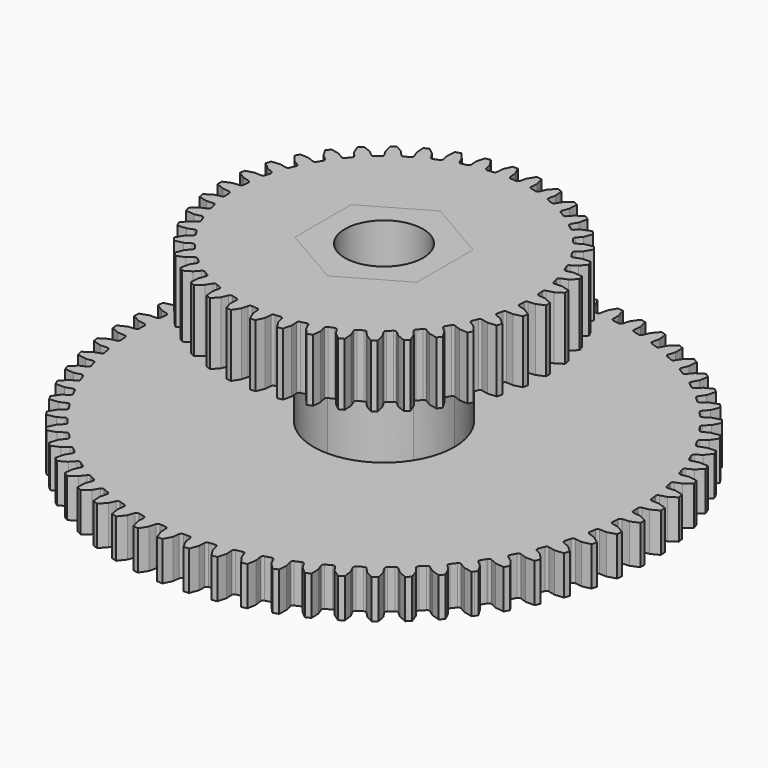
from build123d import *

# Parameters (mm, degrees)
F1_DEPTH = 5
F2_DEPTH = 25
F4_DEPTH = 8
F7_DEPTH = 8


# Not quite as in the source:
# - ends of sketch curves that miss each other by under 0.0002 mm in the source are joined


with BuildPart() as f1:
    # F0 (on Top) → F1 (new body)
    with BuildSketch(Plane.XY):
        with BuildLine():
            ThreePointArc((31.563651726, 1.1618712185), (31.6331481254, 1.3699329355), (31.8224953816, 1.4806896247))
            Line((31.8224953816, 1.4806896247), (32.687195711, 1.6288465021))
            Line((32.687195711, 1.6288465021), (33.6971146214, 2.1645327448))
            ThreePointArc((33.6971146214, 2.1645327448), (33.6729923863, 2.5102054527), (33.6453246363, 2.8556140148))
            Line((33.6453246363, 2.8556140148), (32.5668465724, 3.234789347))
            Line((32.5668465724, 3.234789347), (31.6897239886, 3.2524138587))
            ThreePointArc((31.6897239886, 3.2524138587), (31.4859835528, 3.3337132436), (31.3862532391, 3.5290937234))
            ThreePointArc((31.3862532391, 3.5290937234), (31.3403895973, 3.914224526), (31.2898006773, 4.2987631693))
            ThreePointArc((31.2898006773, 4.2987631693), (31.3382358463, 4.5127039481), (31.515614976, 4.6417634334))
            Line((31.515614976, 4.6417634334), (32.361266405, 4.8752798922))
            Line((32.361266405, 4.8752798922), (33.3128289914, 5.5088604632))
            ThreePointArc((33.3128289914, 5.5088604632), (33.2544100026, 5.8504115039), (33.1924881926, 6.1913487216))
            Line((33.1924881926, 6.1913487216), (32.081616118, 6.4612594425))
            Line((32.081616118, 6.4612594425), (31.2070962224, 6.3914637579))
            ThreePointArc((31.2070962224, 6.3914637579), (30.9962737881, 6.4520724771), (30.8775854889, 6.636551798))
            ThreePointArc((30.8775854889, 6.636551798), (30.7936036369, 7.0152003047), (30.7049784521, 7.3927910806))
            ThreePointArc((30.7049784521, 7.3927910806), (30.7318710291, 7.6104942957), (30.8955184182, 7.7565736913))
            Line((30.8955184182, 7.7565736913), (31.7137165149, 8.0731297672))
            Line((31.7137165149, 8.0731297672), (32.5974668627, 8.7983062647))
            ThreePointArc((32.5974668627, 8.7983062647), (32.5053307694, 9.132341749), (32.409770288, 9.465419392))
            Line((32.409770288, 9.465419392), (31.2775433583, 9.6233833943))
            Line((31.2775433583, 9.6233833943), (30.4143184027, 9.4668605248))
            ThreePointArc((30.4143184027, 9.4668605248), (30.1985089079, 9.506177417), (30.0620422538, 9.6779224586))
            ThreePointArc((30.0620422538, 9.6779224586), (29.9407776219, 10.046324295), (29.8149969133, 10.4132146954))
            ThreePointArc((29.8149969133, 10.4132146954), (29.8200786782, 10.6325166152), (29.9683682449, 10.7941640991))
            Line((29.9683682449, 10.7941640991), (30.7509815902, 11.1906131988))
            Line((30.7509815902, 11.1906131988), (31.5581360159, 12.0001791373))
            ThreePointArc((31.5581360159, 12.0001791373), (31.4331998115, 12.3233780101), (31.3049485598, 12.6452903264))
            Line((31.3049485598, 12.6452903264), (30.1626202609, 12.6897346504))
            Line((30.1626202609, 12.6897346504), (29.3192692462, 12.4480399748))
            ThreePointArc((29.3192692462, 12.4480399748), (29.1006174903, 12.4656739947), (28.9477287795, 12.6229779383))
            ThreePointArc((28.9477287795, 12.6229779383), (28.7903874802, 12.977471585), (28.6287015999, 13.3300146064))
            ThreePointArc((28.6287015999, 13.3300146064), (28.6119215273, 13.548736545), (28.7433791125, 13.7243451593))
            Line((28.7433791125, 13.7243451593), (29.4826297572, 14.1967472867))
            Line((29.4826297572, 14.1967472867), (30.2051661625, 15.08265771))
            ThreePointArc((30.2051661625, 15.08265771), (30.0486646707, 15.3918223554), (29.8890063465, 15.6993503123))
            Line((29.8890063465, 15.6993503123), (28.7479277322, 15.6298383801))
            Line((28.7479277322, 15.6298383801), (27.9328332889, 15.3053740604))
            ThreePointArc((27.9328332889, 15.3053740604), (27.7135115907, 15.3011491618), (27.5457204108, 15.4424489014))
            ThreePointArc((27.5457204108, 15.4424489014), (27.3538656691, 15.7795125157), (27.1578811788, 16.1142052095))
            ThreePointArc((27.1578811788, 16.1142052095), (27.119405043, 16.3301711642), (27.232724466, 16.5179964256))
            Line((27.232724466, 16.5179964256), (27.9212661316, 17.0616567018))
            Line((27.9212661316, 17.0616567018), (28.5520040059, 18.0151061074))
            ThreePointArc((28.5520040059, 18.0151061074), (28.3654989742, 18.3071492684), (28.1760143804, 18.5972518975))
            Line((28.1760143804, 18.5972518975), (27.0475244451, 18.4144727836))
            Line((27.0475244451, 18.4144727836), (26.2687865963, 18.0104649063))
            ThreePointArc((26.2687865963, 18.0104649063), (26.05097685, 17.9844226519), (25.8699495656, 18.1083133484))
            ThreePointArc((25.8699495656, 18.1083133484), (25.6454897503, 18.4245975857), (25.41715473, 18.7381131467))
            ThreePointArc((25.41715473, 18.7381131467), (25.3573650454, 18.9491780499), (25.4514195921, 19.1473526906))
            Line((25.4514195921, 19.1473526906), (26.0824081385, 19.7568687611))
            Line((26.0824081385, 19.7568687611), (26.615079211, 20.7683804544))
            ThreePointArc((26.615079211, 20.7683804544), (26.4004247807, 21.0404002247), (26.1829967881, 21.3101948672))
            Line((26.1829967881, 21.3101948672), (25.0783117692, 21.0159652059))
            Line((25.0783117692, 21.0159652059), (24.343670006, 20.5364274178))
            ThreePointArc((24.343670006, 20.5364274178), (24.1295346822, 20.4888288521), (23.9370720888, 20.5940794569))
            ThreePointArc((23.9370720888, 20.5940794569), (23.6822279221, 20.8864509139), (23.4238217296, 21.1756621721))
            ThreePointArc((23.4238217296, 21.1756621721), (23.3433112218, 21.3797277625), (23.4171666421, 21.5862825685))
            Line((23.4171666421, 21.5862825685), (23.9843317409, 22.2555960356))
            Line((23.9843317409, 22.2555960356), (24.4136423201, 23.3151187565))
            ThreePointArc((24.4136423201, 23.3151187565), (24.1729720167, 23.5644108474), (23.9297615376, 23.8112160983))
            Line((23.9297615376, 23.8112160983), (22.859859219, 23.4084601985))
            Line((22.859859219, 23.4084601985), (22.1766145757, 22.8581583804))
            ThreePointArc((22.1766145757, 22.8581583804), (21.9682829981, 22.7894750221), (21.7662972715, 22.8750393946))
            ThreePointArc((21.7662972715, 22.8750393946), (21.4836103998, 23.1405822351), (21.1976921878, 23.4026273947))
            ThreePointArc((21.1976921878, 23.4026273947), (21.0972619217, 23.5976645972), (21.1501841968, 23.8105467789))
            Line((21.1501841968, 23.8105467789), (21.6478885761, 24.5330054502))
            Line((21.6478885761, 24.5330054502), (21.969570461, 25.6300079217))
            ThreePointArc((21.969570461, 25.6300079217), (21.7052780092, 25.8540965928), (21.4387022173, 26.0754595292))
            Line((21.4387022173, 26.0754595292), (20.414215357, 25.5681792687))
            Line((20.414215357, 25.5681792687), (19.7891587201, 24.9525827024))
            ThreePointArc((19.7891587201, 24.9525827024), (19.5887002497, 24.8634972136), (19.3791981559, 24.9285254092))
            ThreePointArc((19.3791981559, 24.9285254092), (19.0714673403, 25.1646100596), (18.7608659354, 25.3968939925))
            ThreePointArc((18.7608659354, 25.3968939925), (18.6415371851, 25.5809452082), (18.6730006634, 25.798039073))
            Line((18.6730006634, 25.798039073), (19.0962991955, 26.566462448))
            Line((19.0962991955, 26.566462448), (19.3071564304, 27.6900435101))
            ThreePointArc((19.3071564304, 27.6900435101), (19.021867297, 27.8867019467), (18.7345752949, 28.080422713))
            Line((18.7345752949, 28.080422713), (17.7656854476, 27.4736588095))
            Line((17.7656854476, 27.4736588095), (17.2050289822, 26.7988861504))
            ThreePointArc((17.2050289822, 26.7988861504), (17.0144366639, 26.6902842157), (16.799500969, 26.734129471))
            ThreePointArc((16.799500969, 26.734129471), (16.4697950104, 26.938399146), (16.1376088877, 27.1386030268))
            ThreePointArc((16.1376088877, 27.1386030268), (16.0005453544, 27.3098597524), (16.0102365563, 27.5290074775))
            Line((16.0102365563, 27.5290074775), (16.3549213679, 28.3357595699))
            Line((16.3549213679, 28.3357595699), (16.4528582951, 29.4747520795))
            ThreePointArc((16.4528582951, 29.4747520795), (16.1493945917, 29.6420335717), (15.8442271635, 29.8061942989))
            Line((15.8442271635, 29.8061942989), (14.9405924882, 29.1059620557))
            Line((14.9405924882, 29.1059620557), (14.4499072978, 28.3787179535))
            ThreePointArc((14.4499072978, 28.3787179535), (14.2710757289, 28.2516792586), (14.052843003, 28.2739059069))
            ThreePointArc((14.052843003, 28.2739059069), (13.7044390824, 28.4443310479), (13.3539697172, 28.6104650942))
            ThreePointArc((13.3539697172, 28.6104650942), (13.2005333156, 28.7672252925), (13.1883562665, 28.9862489325))
            Line((13.1883562665, 28.9862489325), (13.4510007201, 29.8233117863))
            Line((13.4510007201, 29.8233117863), (13.4350448382, 30.9663948283))
            ThreePointArc((13.4350448382, 30.9663948283), (13.1164357896, 31.1026290805), (12.7964395156, 31.2355892933))
            Line((12.7964395156, 31.2355892933), (11.9670133036, 30.4488650639))
            Line((11.9670133036, 30.4488650639), (11.5511764418, 29.6763778231))
            ThreePointArc((11.5511764418, 29.6763778231), (11.3858822973, 29.5321644588), (11.1665207301, 29.5325520142))
            ThreePointArc((11.1665207301, 29.5325520142), (10.8028825896, 29.6674393791), (10.4376134413, 29.7978523368))
            ThreePointArc((10.4376134413, 29.7978523368), (10.2693284312, 29.9385574456), (10.2354040625, 30.1552796762))
            Line((10.2354040625, 30.1552796762), (10.4133985201, 31.014334165))
            Line((10.4133985201, 31.014334165), (10.2837067176, 32.1501494208))
            ThreePointArc((10.2837067176, 32.1501494208), (9.9531202974, 32.2539816489), (9.6214756139, 32.3544198415))
            Line((9.6214756139, 32.3544198415), (8.8745011338, 31.4890208746))
            Line((8.8745011338, 31.4890208746), (8.5376446929, 30.6789697243))
            ThreePointArc((8.5376446929, 30.6789697243), (8.3875314079, 30.5190145757), (8.1692213306, 30.4975583222))
            ThreePointArc((8.1692213306, 30.4975583222), (7.7939625162, 30.5955683573), (7.4175233491, 30.6889642878))
            ThreePointArc((7.4175233491, 30.6889642878), (7.2360615804, 30.8122152634), (7.1807275432, 31.0244831062))
            Line((7.1807275432, 31.0244831062), (7.2723038742, 31.8969904487))
            Line((7.2723038742, 31.8969904487), (7.0301655467, 33.0142481731))
            ThreePointArc((7.0301655467, 33.0142481731), (6.6908867164, 33.084648628), (6.3508897458, 33.1515665897))
            Line((6.3508897458, 33.1515665897), (5.6937884807, 32.2160945812))
            Line((5.6937884807, 32.2160945812), (5.4392621881, 31.3765275948))
            ThreePointArc((5.4392621881, 31.3765275948), (5.3058203282, 31.2024215924), (5.0907316006, 31.1593357607))
            ThreePointArc((5.0907316006, 31.1593357607), (4.7075831346, 31.2194938198), (4.3237156354, 31.2749444142))
            ThreePointArc((4.3237156354, 31.2749444142), (4.1308793827, 31.3795155239), (4.0546855359, 31.5852195566))
            Line((4.0546855359, 31.5852195566), (4.0589334571, 32.4625094216))
            Line((4.0589334571, 32.4625094216), (3.7067549226, 33.5501058503))
            ThreePointArc((3.7067549226, 33.5501058503), (3.3621395781, 33.5863762806), (3.0171858647, 33.6191073193))
            Line((3.0171858647, 33.6191073193), (2.4564899551, 32.6228578794))
            Line((2.4564899551, 32.6228578794), (2.2868216914, 31.7621202834))
            ThreePointArc((2.2868216914, 31.7621202834), (2.1713787014, 31.5755929654), (1.9616487847, 31.5113054391))
            ThreePointArc((1.9616487847, 31.5113054391), (1.5744167987, 31.5330151281), (1.1869359963, 31.5499693394))
            ThreePointArc((1.1869359963, 31.5499693394), (0.9846437842, 31.6348208181), (0.8883465326, 31.8319159357))
            Line((0.8883465326, 31.8319159357), (0.8052229297, 32.7052690695))
            Line((0.8052229297, 32.7052690695), (0.3465056091, 33.7523955132))
            ThreePointArc((0.3465056091, 33.7523955132), (0.1732483312, 33.7537287976), (0, 33.7541732376))
            Line((0, 33.7541732376), (0, 9))
            ThreePointArc((0, 9), (6.3639610307, 6.3639610307), (9, 0))
            Line((9, 0), (32.5293937768, 0))
            Line((32.5293937768, 0), (31.8574046504, 0.0809088))
            ThreePointArc((31.8574046504, 0.0809088), (31.662771193, 0.1820895238), (31.5829898886, 0.3864290817))
            ThreePointArc((31.5829898886, 0.3864290817), (31.5757012583, 0.7742162854), (31.563651726, 1.1618712185))
        make_face()
        with BuildLine():
            Line((32.728413774, -0.0239623954), (32.5293937768, 0))
            Line((32.5293937768, 0), (9, 0))
            ThreePointArc((9, 0), (8.6444511147, -2.5046885885), (7.6058966832, -4.8114795692))
            Line((7.6058966832, -4.8114795692), (26.6988903909, -16.8896805972))
            ThreePointArc((26.6988903909, -16.8896805972), (26.7200037492, -16.8562324594), (26.7410752039, -16.8227579076))
            ThreePointArc((26.7410752039, -16.8227579076), (26.9157024351, -16.6899954495), (27.1345404693, -16.7051476309))
            Line((27.1345404693, -16.7051476309), (27.9324488599, -17.0698377667))
            Line((27.9324488599, -17.0698377667), (29.0686454276, -17.19614036))
            ThreePointArc((29.0686454276, -17.19614036), (29.2434424406, -16.8969382089), (29.4151519314, -16.5959728227))
            Line((29.4151519314, -16.5959728227), (28.7376717896, -15.6751500926))
            Line((28.7376717896, -15.6751500926), (28.0228863044, -15.1664871314))
            ThreePointArc((28.0228863044, -15.1664871314), (27.9003457013, -14.9845433981), (27.9280062532, -14.7669324738))
            ThreePointArc((27.9280062532, -14.7669324738), (28.1070588783, -14.4228977624), (28.2818785485, -14.076679886))
            ThreePointArc((28.2818785485, -14.076679886), (28.4424212882, -13.9271870312), (28.6616803034, -13.9204745042))
            Line((28.6616803034, -13.9204745042), (29.4919339783, -14.2039059783))
            Line((29.4919339783, -14.2039059783), (30.6350606582, -14.2164518711))
            ThreePointArc((30.6350606582, -14.2164518711), (30.7791973484, -13.9013356907), (30.9200869136, -13.5847696343))
            Line((30.9200869136, -13.5847696343), (30.1542895803, -12.7359752265))
            Line((30.1542895803, -12.7359752265), (29.3924105022, -12.3010083459))
            ThreePointArc((29.3924105022, -12.3010083459), (29.2523634991, -12.1321701839), (29.2582194203, -11.9128869892))
            ThreePointArc((29.2582194203, -11.9128869892), (29.4021261258, -11.5527363162), (29.5416050041, -11.1908323064))
            ThreePointArc((29.5416050041, -11.1908323064), (29.6864657831, -11.0260945816), (29.9039669872, -10.9975844778))
            Line((29.9039669872, -10.9975844778), (30.7583169113, -11.1969406925))
            Line((30.7583169113, -11.1969406925), (31.8970112286, -11.0956062441))
            ThreePointArc((31.8970112286, -11.0956062441), (32.009055333, -10.767707368), (32.1177252638, -10.4386855828))
            Line((32.1177252638, -10.4386855828), (31.2712220986, -9.6703554246))
            Line((31.2712220986, -9.6703554246), (30.469819562, -9.3134089313))
            ThreePointArc((30.469819562, -9.3134089313), (30.3136574479, -9.15935455), (30.2976506063, -8.9405772593))
            ThreePointArc((30.2976506063, -8.9405772593), (30.4049865194, -8.5678756466), (30.5077340259, -8.1938977323))
            ThreePointArc((30.5077340259, -8.1938977323), (30.635473864, -8.0155522387), (30.8490556186, -7.9655274045))
            Line((30.8490556186, -7.9655274045), (31.7190081283, -8.0788265895))
            Line((31.7190081283, -8.0788265895), (32.8419554021, -7.8646185883))
            ThreePointArc((32.8419554021, -7.8646185883), (32.9207943845, -7.527192964), (32.996165117, -7.188982447))
            Line((32.996165117, -7.188982447), (32.0773666189, -6.5087582443))
            Line((32.0773666189, -6.5087582443), (31.2444066165, -6.2333792754))
            ThreePointArc((31.2444066165, -6.2333792754), (31.0736809024, -6.0956389641), (31.0359710383, -5.8795424546))
            ThreePointArc((31.0359710383, -5.8795424546), (31.1056634342, -5.4980097268), (31.1706643195, -5.1156592853))
            ThreePointArc((31.1706643195, -5.1156592853), (31.2800118942, -4.9254782333), (31.4875517324, -4.8544365638))
            Line((31.4875517324, -4.8544365638), (32.3644623607, -4.8805538426))
            Line((32.3644623607, -4.8805538426), (33.4605016817, -4.5556001551))
            ThreePointArc((33.4605016817, -4.5556001551), (33.505351054, -4.2120068637), (33.5466723525, -3.867973006))
            Line((33.5466723525, -3.867973006), (32.5647114329, -3.2826060821))
            Line((32.5647114329, -3.2826060821), (31.7084716564, -3.0915323954))
            ThreePointArc((31.7084716564, -3.0915323954), (31.52488042, -2.971475066), (31.4658415873, -2.7602076411))
            ThreePointArc((31.4658415873, -2.7602076411), (31.497200057, -2.3736182666), (31.523808944, -1.9866803216))
            ThreePointArc((31.523808944, -1.9866803216), (31.6136753387, -1.7865851362), (31.8131101742, -1.6952319844))
            Line((31.8131101742, -1.6952319844), (32.6882648392, -1.6339074581))
            Line((32.6882648392, -1.6339074581), (33.7465012814, -1.201438327))
            ThreePointArc((33.7465012814, -1.201438327), (33.7569175718, -0.8550884816), (33.7637788438, -0.5086499748))
            Line((33.7637788438, -0.5086499748), (32.728413774, -0.0239623954))
        make_face()
        with BuildLine():
            Line((26.6988903909, -16.8896805972), (7.6058966832, -4.8114795692))
            ThreePointArc((7.6058966832, -4.8114795692), (4.3414677171, -7.8836322886), (0, -9))
            Line((0, -9), (0, -31.5987587334))
            ThreePointArc((0, -31.5987587334), (0.1939231563, -31.5981634204), (0.3878390027, -31.5963775036))
            ThreePointArc((0.3878390027, -31.5963775036), (0.5941060189, -31.6710388551), (0.7001078112, -31.8630889696))
            Line((0.7001078112, -31.8630889696), (0.8266605616, -32.7312138718))
            Line((0.8266605616, -32.7312138718), (1.3370035814, -33.7541732376))
            ThreePointArc((1.3370035814, -33.7541732376), (1.6831759783, -33.7386771015), (2.0291545231, -33.7196299133))
            Line((2.0291545231, -33.7196299133), (2.4351053121, -32.6509398992))
            Line((2.4351053121, -32.6509398992), (2.4745924056, -31.7745279895))
            ThreePointArc((2.4745924056, -31.7745279895), (2.560944869, -31.5728784258), (2.7587508585, -31.4780496064))
            ThreePointArc((2.7587508585, -31.4780496064), (3.144893984, -31.4418040065), (3.5305742805, -31.4008177806))
            ThreePointArc((3.5305742805, -31.4008177806), (3.7432527735, -31.454571095), (3.8678495127, -31.635112178))
            Line((3.8678495127, -31.635112178), (4.0802110834, -32.4863222014))
            Line((4.0802110834, -32.4863222014), (4.6898718579, -33.45338455))
            ThreePointArc((4.6898718579, -33.45338455), (5.0327774527, -33.4034981633), (5.3751405473, -33.3500972784))
            Line((5.3751405473, -33.3500972784), (5.672669821, -32.2462971945))
            Line((5.672669821, -32.2462971945), (5.6246982753, -31.3703091958))
            ThreePointArc((5.6246982753, -31.3703091958), (5.6905439596, -31.1610634847), (5.8779257032, -31.0470110467))
            ThreePointArc((5.8779257032, -31.0470110467), (6.2585372526, -30.9724987959), (6.6382204255, -30.8933148594))
            ThreePointArc((6.6382204255, -30.8933148594), (6.855197782, -30.9256242445), (6.9971516309, -31.0928625417))
            Line((6.9971516309, -31.0928625417), (7.2932105784, -31.9186982198))
            Line((7.2932105784, -31.9186982198), (7.9961296752, -32.8202528259))
            ThreePointArc((7.9961296752, -32.8202528259), (8.3323614028, -32.73647246), (8.6677064176, -32.6492485587))
            Line((8.6677064176, -32.6492485587), (8.8538572958, -31.5213087556))
            Line((8.8538572958, -31.5213087556), (8.7189040108, -30.6544504263))
            ThreePointArc((8.7189040108, -30.6544504263), (8.7635880127, -30.4396877691), (8.9386820844, -30.3075448293))
            ThreePointArc((8.9386820844, -30.3075448293), (9.3099958748, -30.1955025168), (9.6798924797, -30.0789127085))
            ThreePointArc((9.6798924797, -30.0789127085), (9.899012038, -30.0894562751), (10.056912031, -30.2417296467))
            Line((10.056912031, -30.2417296467), (10.4337275418, -31.0339836825))
            Line((10.4337275418, -31.0339836825), (11.2229187428, -31.861070233))
            ThreePointArc((11.2229187428, -31.861070233), (11.5491351896, -31.7442290432), (11.8741290503, -31.6240490469))
            Line((11.8741290503, -31.6240490469), (11.9470510479, -30.4831779507))
            Line((11.9470510479, -30.4831779507), (11.7264573691, -29.6340646569))
            ThreePointArc((11.7264573691, -29.6340646569), (11.7495360451, -29.4159202133), (11.9106030267, -29.26700042))
            ThreePointArc((11.9106030267, -29.26700042), (12.2689125212, -29.1185450059), (12.6253625529, -28.9657047374))
            ThreePointArc((12.6253625529, -28.9657047374), (12.844445638, -28.9543772609), (13.0167225757, -29.0901724852))
            Line((13.0167225757, -29.0901724852), (13.4705484159, -29.8409705849))
            Line((13.4705484159, -29.8409705849), (14.3381693691, -30.585368533))
            ThreePointArc((14.3381693691, -30.585368533), (14.651127867, -30.4366297136), (14.9625404001, -30.2846881687))
            Line((14.9625404001, -30.2846881687), (14.9215092243, -29.1422241014))
            Line((14.9215092243, -29.1422241014), (14.617467436, -28.3192945793))
            ThreePointArc((14.617467436, -28.3192945793), (14.6187120131, -28.0999358541), (14.7641512167, -27.9357189926))
            ThreePointArc((14.7641512167, -27.9357189926), (15.1059095636, -27.7523187582), (15.4453840208, -27.564739171))
            ThreePointArc((15.4453840208, -27.564739171), (15.662225808, -27.5316686218), (15.8471676948, -27.6496357409))
            Line((15.8471676948, -27.6496357409), (16.3734924061, -28.3515159644))
            Line((16.3734924061, -28.3515159644), (17.3109204729, -29.0058286881))
            ThreePointArc((17.3109204729, -29.0058286881), (17.6075115542, -28.8266696204), (17.9022484327, -28.6444762761))
            Line((17.9022484327, -28.6444762761), (17.747671312, -27.5117733875))
            Line((17.747671312, -27.5117733875), (17.3632028185, -26.723205585))
            ThreePointArc((17.3632028185, -26.723205585), (17.3425994701, -26.5048128414), (17.4709653106, -26.3269306141))
            ThreePointArc((17.4709653106, -26.3269306141), (17.7927626163, -26.1104159538), (18.1118734798, -25.8899676402))
            ThreePointArc((18.1118734798, -25.8899676402), (18.3243470913, -25.8354690606), (18.5201152717, -25.9344348502))
            Line((18.5201152717, -25.9344348502), (19.1137107127, -26.5804234551))
            Line((19.1137107127, -26.5804234551), (20.111628165, -27.1381468311))
            ThreePointArc((20.111628165, -27.1381468311), (20.3889182023, -26.9303387363), (20.6640631821, -26.7196939516))
            Line((20.6640631821, -26.7196939516), (20.3974490571, -25.6080289722))
            Line((20.3974490571, -25.6080289722), (19.9363752906, -24.8616610852))
            ThreePointArc((19.9363752906, -24.8616610852), (19.8941298282, -24.6464053924), (20.0041455949, -24.456626221))
            ThreePointArc((20.0041455949, -24.456626221), (20.3027833423, -24.209148395), (20.5983590021, -23.9580223325))
            ThreePointArc((20.5983590021, -23.9580223325), (20.8043535444, -23.8826372628), (21.0090024533, -23.9616197434))
            Line((21.0090024533, -23.9616197434), (21.6639670598, -24.5452947106))
            Line((21.6639670598, -24.5452947106), (22.712457707, -25.0008856882))
            ThreePointArc((22.712457707, -25.0008856882), (22.9676756722, -24.7665037101), (23.2204797018, -24.5295103634))
            Line((23.2204797018, -24.5295103634), (22.8445080335, -23.4499130749))
            Line((22.8445080335, -23.4499130749), (22.3114099331, -22.7531614663))
            ThreePointArc((22.3114099331, -22.7531614663), (22.247941956, -22.5431817693), (22.338515783, -22.3433917976))
            ThreePointArc((22.338515783, -22.3433917976), (22.6110265697, -22.067411311), (22.8801292159, -21.7881035321))
            ThreePointArc((22.8801292159, -21.7881035321), (23.0775957771, -21.6925798894), (23.2890925247, -21.7507934833))
            Line((23.2890925247, -21.7507934833), (23.9989182244, -22.266354853))
            Line((23.9989182244, -22.266354853), (25.0875609234, -22.6152854818))
            ThreePointArc((25.0875609234, -22.6152854818), (25.3181711293, -22.3566596359), (25.5461223345, -22.0956724761))
            Line((25.5461223345, -22.0956724761), (25.0645273916, -21.0588726785))
            Line((25.0645273916, -21.0588726785), (24.4647048828, -20.4186622656))
            ThreePointArc((24.4647048828, -20.4186622656), (24.3806449522, -20.2160456399), (24.4508758857, -20.0082303148))
            ThreePointArc((24.4508758857, -20.0082303148), (24.694551739, -19.706490352), (24.9345070183, -19.4017766856))
            ThreePointArc((24.9345070183, -19.4017766856), (25.1214838326, -19.2870637982), (25.3377256906, -19.3239296856))
            Line((25.3377256906, -19.3239296856), (26.0953571622, -19.766252985))
            Line((26.0953571622, -19.766252985), (27.2133317948, -20.005056131))
            ThreePointArc((27.2133317948, -20.005056131), (27.3023879135, -19.8832627697), (27.3909062414, -19.7610612959))
            ThreePointArc((27.3909062414, -19.7610612959), (27.5048526856, -19.6020446961), (27.6178759782, -19.4423706328))
            Line((27.6178759782, -19.4423706328), (27.0354450622, -18.4586706909))
            Line((27.0354450622, -18.4586706909), (26.3748588726, -17.8813653322))
            ThreePointArc((26.3748588726, -17.8813653322), (26.271042222, -17.6881251038), (26.3202323987, -17.474349458))
            ThreePointArc((26.3202323987, -17.474349458), (26.5111708995, -17.1830627377), (26.6988903909, -16.8896805972))
        make_face()
        with BuildLine():
            Line((0, -31.5987587334), (0, -9))
            ThreePointArc((0, -9), (-6.3618979129, -6.3660234798), (-8.9999981089, -0.0058344324))
            Line((-8.9999981089, -0.0058344324), (-32.7054872674, -0.0212019993))
            Line((-32.7054872674, -0.0212019993), (-32.728413774, -0.0239623954))
            Line((-32.728413774, -0.0239623954), (-33.763778768, -0.5086421812))
            ThreePointArc((-33.763778768, -0.5086421812), (-33.7569177729, -0.8550804174), (-33.7465021104, -1.2014268906))
            Line((-33.7465021104, -1.2014268906), (-32.6882648392, -1.6339074581))
            Line((-32.6882648392, -1.6339074581), (-31.8131101163, -1.6952311584))
            ThreePointArc((-31.8131101163, -1.6952311584), (-31.613675704, -1.7865847682), (-31.5238077529, -1.986692715))
            ThreePointArc((-31.5238077529, -1.986692715), (-31.4971984994, -2.3736390515), (-31.465840077, -2.7602211069))
            ThreePointArc((-31.465840077, -2.7602211069), (-31.52488042, -2.971475066), (-31.7084716505, -3.0915324217))
            Line((-31.7084716505, -3.0915324217), (-32.5647114329, -3.2826060821))
            Line((-32.5647114329, -3.2826060821), (-33.5466730032, -3.8679667871))
            ThreePointArc((-33.5466730032, -3.8679667871), (-33.5053522603, -4.2119972383), (-33.4605034208, -4.5555855631))
            Line((-33.4605034208, -4.5555855631), (-32.3644623607, -4.8805538426))
            Line((-32.3644623607, -4.8805538426), (-31.4875517324, -4.8544365668))
            ThreePointArc((-31.4875517324, -4.8544365668), (-31.2800118942, -4.9254782333), (-31.170666204, -5.1156445376))
            ThreePointArc((-31.170666204, -5.1156445376), (-31.1056626192, -5.4980143491), (-31.0359689743, -5.8795528472))
            ThreePointArc((-31.0359689743, -5.8795528472), (-31.0736812105, -6.0956394871), (-31.2444064691, -6.2333797213))
            Line((-31.2444064691, -6.2333797213), (-32.0773666189, -6.5087582443))
            Line((-32.0773666189, -6.5087582443), (-32.9961654636, -7.1889825224))
            ThreePointArc((-32.9961654636, -7.1889825224), (-32.9207924533, -7.527201425), (-32.8419521118, -7.8646330928))
            Line((-32.8419521118, -7.8646330928), (-31.7190081283, -8.0788265895))
            Line((-31.7190081283, -8.0788265895), (-30.849054626, -7.9655270478))
            ThreePointArc((-30.849054626, -7.9655270478), (-30.6354738529, -8.0155522462), (-30.5077377694, -8.1938854323))
            ThreePointArc((-30.5077377694, -8.1938854323), (-30.4049853207, -8.567879907), (-30.2976489543, -8.9405836188))
            ThreePointArc((-30.2976489543, -8.9405836188), (-30.313657249, -9.1593541192), (-30.469819631, -9.3134087765))
            Line((-30.469819631, -9.3134087765), (-31.2712220986, -9.6703554246))
            Line((-31.2712220986, -9.6703554246), (-32.1177264701, -10.4386814811))
            ThreePointArc((-32.1177264701, -10.4386814811), (-32.0090535541, -10.7677126627), (-31.897007696, -11.0956175287))
            Line((-31.897007696, -11.0956175287), (-30.7583169113, -11.1969406925))
            Line((-30.7583169113, -11.1969406925), (-29.9039670709, -10.9975841191))
            ThreePointArc((-29.9039670709, -10.9975841191), (-29.6864657831, -11.0260945816), (-29.541607648, -11.1908238154))
            ThreePointArc((-29.541607648, -11.1908238154), (-29.4021299707, -11.5527265195), (-29.2582177314, -11.9128908808))
            ThreePointArc((-29.2582177314, -11.9128908808), (-29.2523634991, -12.1321701839), (-29.3924107486, -12.3010079142))
            Line((-29.3924107486, -12.3010079142), (-30.1542895803, -12.7359752265))
            Line((-30.1542895803, -12.7359752265), (-30.9200877564, -13.5847685092))
            ThreePointArc((-30.9200877564, -13.5847685092), (-30.7791952442, -13.9013403542), (-30.6350572345, -14.2164600409))
            Line((-30.6350572345, -14.2164600409), (-29.4919339783, -14.2039059783))
            Line((-29.4919339783, -14.2039059783), (-28.661680564, -13.9204737411))
            ThreePointArc((-28.661680564, -13.9204737411), (-28.4424212882, -13.9271870312), (-28.2818814167, -14.0766745673))
            ThreePointArc((-28.2818814167, -14.0766745673), (-28.1070639676, -14.4228878354), (-27.9280061137, -14.7669334391))
            ThreePointArc((-27.9280061137, -14.7669334391), (-27.9003457013, -14.9845433981), (-28.0228866836, -15.1664865986))
            Line((-28.0228866836, -15.1664865986), (-28.7376717896, -15.6751500926))
            Line((-28.7376717896, -15.6751500926), (-29.4151510367, -16.5959749821))
            ThreePointArc((-29.4151510367, -16.5959749821), (-29.2434398623, -16.8969426746), (-29.0686425345, -17.1961446483))
            Line((-29.0686425345, -17.1961446483), (-27.9324488599, -17.0698377667))
            Line((-27.9324488599, -17.0698377667), (-27.1345404714, -16.7051476264))
            ThreePointArc((-27.1345404714, -16.7051476264), (-26.9157024351, -16.6899954495), (-26.7410759781, -16.8227556631))
            ThreePointArc((-26.7410759781, -16.8227556631), (-26.5326577524, -17.1498402434), (-26.3202339142, -17.4743476961))
            ThreePointArc((-26.3202339142, -17.4743476961), (-26.271042222, -17.6881251038), (-26.3748587984, -17.8813654172))
            Line((-26.3748587984, -17.8813654172), (-27.0354450622, -18.4586706909))
            Line((-27.0354450622, -18.4586706909), (-27.6178726777, -19.4423746597))
            ThreePointArc((-27.6178726777, -19.4423746597), (-27.4170407659, -19.7247611564), (-27.2133310482, -20.0050584238))
            Line((-27.2133310482, -20.0050584238), (-26.0953571622, -19.766252985))
            Line((-26.0953571622, -19.766252985), (-25.3377255052, -19.3239300032))
            ThreePointArc((-25.3377255052, -19.3239300032), (-25.1214838326, -19.2870637982), (-24.9345066406, -19.4017771998))
            ThreePointArc((-24.9345066406, -19.4017771998), (-24.6945586744, -19.7064816553), (-24.450879903, -20.0082260453))
            ThreePointArc((-24.450879903, -20.0082260453), (-24.3806449522, -20.2160456399), (-24.4647047673, -20.4186623738))
            Line((-24.4647047673, -20.4186623738), (-25.0645273916, -21.0588726785))
            Line((-25.0645273916, -21.0588726785), (-25.5461161604, -22.0956787618))
            ThreePointArc((-25.5461161604, -22.0956787618), (-25.3181679605, -22.3566632267), (-25.0875620957, -22.615284563))
            Line((-25.0875620957, -22.615284563), (-23.9989182244, -22.266354853))
            Line((-23.9989182244, -22.266354853), (-23.2890929124, -21.7507929495))
            ThreePointArc((-23.2890929124, -21.7507929495), (-23.0775957771, -21.6925798894), (-22.8801258118, -21.7881063758))
            ThreePointArc((-22.8801258118, -21.7881063758), (-22.6110340131, -22.0674036796), (-22.3385218102, -22.3433863956))
            ThreePointArc((-22.3385218102, -22.3433863956), (-22.2479419352, -22.5431820843), (-22.3114103495, -22.7531619427))
            Line((-22.3114103495, -22.7531619427), (-22.8445080335, -23.4499130749))
            Line((-22.8445080335, -23.4499130749), (-23.2204712948, -24.5295185752))
            ThreePointArc((-23.2204712948, -24.5295185752), (-22.9676721879, -24.7665069431), (-22.7124617127, -25.0008824059))
            Line((-22.7124617127, -25.0008824059), (-21.6639670598, -24.5452947106))
            Line((-21.6639670598, -24.5452947106), (-21.0090028848, -23.9616192593))
            ThreePointArc((-21.0090028848, -23.9616192593), (-20.8043528119, -23.8826372564), (-20.5983527765, -23.9580275373))
            ThreePointArc((-20.5983527765, -23.9580275373), (-20.3027796712, -24.2091514754), (-20.0041548828, -24.4566191015))
            ThreePointArc((-20.0041548828, -24.4566191015), (-19.8941298282, -24.6464053924), (-19.9363757842, -24.8616607802))
            Line((-19.9363757842, -24.8616607802), (-20.3974490571, -25.6080289722))
            Line((-20.3974490571, -25.6080289722), (-20.6640505767, -26.719703125))
            ThreePointArc((-20.6640505767, -26.719703125), (-20.3889140604, -26.9303418737), (-20.1116356237, -27.1381418866))
            Line((-20.1116356237, -27.1381418866), (-19.1137107127, -26.5804234551))
            Line((-19.1137107127, -26.5804234551), (-18.5201159539, -25.934435178))
            ThreePointArc((-18.5201159539, -25.934435178), (-18.3243474407, -25.8354690987), (-18.1118649248, -25.889973527))
            ThreePointArc((-18.1118649248, -25.889973527), (-17.7927586792, -26.1104186381), (-17.4709782463, -26.3269230067))
            ThreePointArc((-17.4709782463, -26.3269230067), (-17.3425994701, -26.5048128414), (-17.3632028922, -26.723205549))
            Line((-17.3632028922, -26.723205549), (-17.747671312, -27.5117733875))
            Line((-17.747671312, -27.5117733875), (-17.9022606075, -28.6444685342))
            ThreePointArc((-17.9022606075, -28.6444685342), (-17.6075218924, -28.8266633029), (-17.3109310519, -29.0058227707))
            Line((-17.3109310519, -29.0058227707), (-16.3734924061, -28.3515159644))
            Line((-16.3734924061, -28.3515159644), (-15.8471675293, -27.649634826))
            ThreePointArc((-15.8471675293, -27.649634826), (-15.6622254013, -27.5316685359), (-15.4453718659, -27.5647459636))
            ThreePointArc((-15.4453718659, -27.5647459636), (-15.1058909999, -27.7523288675), (-14.7641384663, -27.9357257315))
            ThreePointArc((-14.7641384663, -27.9357257315), (-14.6187118491, -28.0999362831), (-14.6174677989, -28.3192944452))
            Line((-14.6174677989, -28.3192944452), (-14.9215092243, -29.1422241014))
            Line((-14.9215092243, -29.1422241014), (-14.9625506578, -30.2846827061))
            ThreePointArc((-14.9625506578, -30.2846827061), (-14.6511383313, -30.4366246742), (-14.3381831236, -30.5853628268))
            Line((-14.3381831236, -30.5853628268), (-13.4705484159, -29.8409705849))
            Line((-13.4705484159, -29.8409705849), (-13.0167226947, -29.0901724133))
            ThreePointArc((-13.0167226947, -29.0901724133), (-12.844445638, -28.9543772609), (-12.6253759677, -28.965698292))
            ThreePointArc((-12.6253759677, -28.965698292), (-12.2689084413, -29.1185467258), (-11.9105937375, -29.2670047277))
            ThreePointArc((-11.9105937375, -29.2670047277), (-11.7495360451, -29.4159202133), (-11.7264570317, -29.6340647445))
            Line((-11.7264570317, -29.6340647445), (-11.9470510479, -30.4831779507))
            Line((-11.9470510479, -30.4831779507), (-11.8741362934, -31.6240458504))
            ThreePointArc((-11.8741362934, -31.6240458504), (-11.5491299398, -31.744230954), (-11.2229041437, -31.8610752774))
            Line((-11.2229041437, -31.8610752774), (-10.4337275418, -31.0339836825))
            Line((-10.4337275418, -31.0339836825), (-10.0569123027, -30.2417295175))
            ThreePointArc((-10.0569123027, -30.2417295175), (-9.899012038, -30.0894562751), (-9.6799039866, -30.0789087947))
            ThreePointArc((-9.6799039866, -30.0789087947), (-9.3099913077, -30.1955039255), (-8.9386760156, -30.3075474669))
            ThreePointArc((-8.9386760156, -30.3075474669), (-8.7635880127, -30.4396877691), (-8.7189038093, -30.6544504577))
            Line((-8.7189038093, -30.6544504577), (-8.8538572958, -31.5213087556))
            Line((-8.8538572958, -31.5213087556), (-8.6677105345, -32.6492473725))
            ThreePointArc((-8.6677105345, -32.6492473725), (-8.3323567643, -32.7364736411), (-7.9961182009, -32.8202557571))
            Line((-7.9961182009, -32.8202557571), (-7.2932105784, -31.9186982198))
            Line((-7.2932105784, -31.9186982198), (-6.9971514066, -31.0928626221))
            ThreePointArc((-6.9971514066, -31.0928626221), (-6.855197782, -30.9256242445), (-6.6382288105, -30.8933131211))
            ThreePointArc((-6.6382288105, -30.8933131211), (-6.2585481378, -30.9724965954), (-5.8779218024, -31.0470123941))
            ThreePointArc((-5.8779218024, -31.0470123941), (-5.6905442794, -31.1610630763), (-5.62469809, -31.3703092059))
            Line((-5.62469809, -31.3703092059), (-5.672669821, -32.2462971945))
            Line((-5.672669821, -32.2462971945), (-5.375142546, -33.3500967866))
            ThreePointArc((-5.375142546, -33.3500967866), (-5.0327722977, -33.4034989403), (-4.6898625927, -33.4533862012))
            Line((-4.6898625927, -33.4533862012), (-4.0802110834, -32.4863222014))
            Line((-4.0802110834, -32.4863222014), (-3.8678493804, -31.635112211))
            ThreePointArc((-3.8678493804, -31.635112211), (-3.7432527735, -31.454571095), (-3.5305794178, -31.4008172683))
            ThreePointArc((-3.5305794178, -31.4008172683), (-3.1449043731, -31.4418029669), (-2.758749888, -31.4780503876))
            ThreePointArc((-2.758749888, -31.4780503876), (-2.5609452281, -31.5728780511), (-2.4745924461, -31.7745279913))
            Line((-2.4745924461, -31.7745279913), (-2.4351053121, -32.6509398992))
            Line((-2.4351053121, -32.6509398992), (-2.0291524318, -33.7196296935))
            ThreePointArc((-2.0291524318, -33.7196296935), (-1.6831708186, -33.738677359), (-1.3369973776, -33.7541739982))
            Line((-1.3369973776, -33.7541739982), (-0.8266605616, -32.7312138718))
            Line((-0.8266605616, -32.7312138718), (-0.70010757, -31.8630890048))
            ThreePointArc((-0.70010757, -31.8630890048), (-0.5941060189, -31.6710388551), (-0.387841074, -31.5963769574))
            ThreePointArc((-0.387841074, -31.5963769574), (-0.1939288703, -31.5981633853), (0, -31.5987587334))
        make_face()
        with BuildLine():
            ThreePointArc((-8.9999981089, -0.0058344324), (-8.6452625182, 2.5018864865), (-7.6058966832, 4.8114795692))
            Line((-7.6058966832, 4.8114795692), (-28.5308450917, 18.0485725703))
            ThreePointArc((-28.5308450917, 18.0485725703), (-28.5414290638, 18.0318430412), (-28.5520032263, 18.0151073101))
            Line((-28.5520032263, 18.0151073101), (-27.9212661316, 17.0616567018))
            Line((-27.9212661316, 17.0616567018), (-27.2327246799, 16.5179961546))
            ThreePointArc((-27.2327246799, 16.5179961546), (-27.119405043, 16.3301711642), (-27.1578783474, 16.1142095351))
            ThreePointArc((-27.1578783474, 16.1142095351), (-27.3538555512, 15.7795300404), (-27.5457158517, 15.4424559482))
            ThreePointArc((-27.5457158517, 15.4424559482), (-27.7135120456, 15.3011490007), (-27.9328333746, 15.3053738451))
            Line((-27.9328333746, 15.3053738451), (-28.7479277322, 15.6298383801))
            Line((-28.7479277322, 15.6298383801), (-29.8890075874, 15.6993483404))
            ThreePointArc((-29.8890075874, 15.6993483404), (-30.0486699697, 15.3918120194), (-30.205164139, 15.0826618932))
            Line((-30.205164139, 15.0826618932), (-29.4826297572, 14.1967472867))
            Line((-29.4826297572, 14.1967472867), (-28.7433790019, 13.7243453323))
            ThreePointArc((-28.7433790019, 13.7243453323), (-28.6119215273, 13.548736545), (-28.6287004248, 13.3300176599))
            ThreePointArc((-28.6287004248, 13.3300176599), (-28.7903853756, 12.9774762493), (-28.9477240432, 12.6229885285))
            ThreePointArc((-28.9477240432, 12.6229885285), (-29.1006174903, 12.4656739947), (-29.3192691384, 12.4480403512))
            Line((-29.3192691384, 12.4480403512), (-30.1626202609, 12.6897346504))
            Line((-30.1626202609, 12.6897346504), (-31.3049510688, 12.6452853057))
            ThreePointArc((-31.3049510688, 12.6452853057), (-31.4331979439, 12.3233827688), (-31.5581329423, 12.0001874658))
            Line((-31.5581329423, 12.0001874658), (-30.7509815902, 11.1906131988))
            Line((-30.7509815902, 11.1906131988), (-29.9683682813, 10.7941640271))
            ThreePointArc((-29.9683682813, 10.7941640271), (-29.8200786782, 10.6325166152), (-29.8149973217, 10.4132134359))
            ThreePointArc((-29.8149973217, 10.4132134359), (-29.9407760549, 10.0463289592), (-30.0620372774, 9.6779370751))
            ThreePointArc((-30.0620372774, 9.6779370751), (-30.1985089079, 9.506177417), (-30.414318346, 9.4668608375))
            Line((-30.414318346, 9.4668608375), (-31.2775433583, 9.6233833943))
            Line((-31.2775433583, 9.6233833943), (-32.4097719952, 9.4654152795))
            ThreePointArc((-32.4097719952, 9.4654152795), (-32.5053294355, 9.1323464899), (-32.5974637782, 8.7983177024))
            Line((-32.5974637782, 8.7983177024), (-31.7137165149, 8.0731297672))
            Line((-31.7137165149, 8.0731297672), (-30.8955185865, 7.7565732561))
            ThreePointArc((-30.8955185865, 7.7565732561), (-30.7318710291, 7.6104942957), (-30.7049794686, 7.3927869192))
            ThreePointArc((-30.7049794686, 7.3927869192), (-30.7936059937, 7.0151899792), (-30.8775878599, 6.6365393931))
            ThreePointArc((-30.8775878599, 6.6365393931), (-30.9962737881, 6.4520724771), (-31.207096231, 6.391463651))
            Line((-31.207096231, 6.391463651), (-32.081616118, 6.4612594425))
            Line((-32.081616118, 6.4612594425), (-33.1924892038, 6.1913424824))
            ThreePointArc((-33.1924892038, 6.1913424824), (-33.2544088608, 5.850417979), (-33.3128269485, 5.508875015))
            Line((-33.3128269485, 5.508875015), (-32.361266405, 4.8752798922))
            Line((-32.361266405, 4.8752798922), (-31.5156160892, 4.6417631646))
            ThreePointArc((-31.5156160892, 4.6417631646), (-31.3382361216, 4.5127043664), (-31.2898012505, 4.2987558321))
            ThreePointArc((-31.2898012505, 4.2987558321), (-31.340390904, 3.9142140989), (-31.3862540494, 3.5290833076))
            ThreePointArc((-31.3862540494, 3.5290833076), (-31.4859835528, 3.3337132436), (-31.689724, 3.2524144272))
            Line((-31.689724, 3.2524144272), (-32.5668465724, 3.234789347))
            Line((-32.5668465724, 3.234789347), (-33.6453257995, 2.855606233))
            ThreePointArc((-33.6453257995, 2.855606233), (-33.6729930447, 2.510196667), (-33.6971151105, 2.1645171914))
            Line((-33.6971151105, 2.1645171914), (-32.687195711, 1.6288465021))
            Line((-32.687195711, 1.6288465021), (-31.8224964182, 1.480689639))
            ThreePointArc((-31.8224964182, 1.480689639), (-31.6331484482, 1.3699333331), (-31.563651726, 1.1618712185))
            ThreePointArc((-31.563651726, 1.1618712185), (-31.5757015306, 0.774205364), (-31.5829901647, 0.3864218122))
            ThreePointArc((-31.5829901647, 0.3864218122), (-31.662771193, 0.1820895238), (-31.8574046583, 0.0809088655))
            Line((-31.8574046583, 0.0809088655), (-32.7054872674, -0.0212019993))
            Line((-32.7054872674, -0.0212019993), (-8.9999981089, -0.0058344324))
        make_face()
        with BuildLine():
            ThreePointArc((-7.6058966832, 4.8114795692), (-4.3414677171, 7.8836322886), (0, 9))
            Line((0, 9), (0, 33.7541732376))
            ThreePointArc((0, 33.7541732376), (-0.1732545648, 33.7537287656), (-0.3465045685, 33.7523953612))
            Line((-0.3465045685, 33.7523953612), (-0.8052229297, 32.7052690695))
            Line((-0.8052229297, 32.7052690695), (-0.888345833, 31.831915968))
            ThreePointArc((-0.888345833, 31.831915968), (-0.984643371, 31.6348212083), (-1.1869298039, 31.5499704445))
            ThreePointArc((-1.1869298039, 31.5499704445), (-1.5743965058, 31.5330161409), (-1.9616404107, 31.5113054806))
            ThreePointArc((-1.9616404107, 31.5113054806), (-2.1713787014, 31.5755929654), (-2.2868216892, 31.7621202838))
            Line((-2.2868216892, 31.7621202838), (-2.4564899551, 32.6228578794))
            Line((-2.4564899551, 32.6228578794), (-3.0171879805, 33.6191077409))
            ThreePointArc((-3.0171879805, 33.6191077409), (-3.3621509961, 33.586375138), (-3.7067506708, 33.5501060222))
            Line((-3.7067506708, 33.5501060222), (-4.0589334571, 32.4625094216))
            Line((-4.0589334571, 32.4625094216), (-4.054684997, 31.5852195592))
            ThreePointArc((-4.054684997, 31.5852195592), (-4.1308793827, 31.3795155239), (-4.3237125927, 31.274944952))
            ThreePointArc((-4.3237125927, 31.274944952), (-4.7075779056, 31.2194946079), (-5.0907200691, 31.1593372113))
            ThreePointArc((-5.0907200691, 31.1593372113), (-5.3058203282, 31.2024215924), (-5.4392616895, 31.376527746))
            Line((-5.4392616895, 31.376527746), (-5.6937884807, 32.2160945812))
            Line((-5.6937884807, 32.2160945812), (-6.3508950682, 33.151566216))
            ThreePointArc((-6.3508950682, 33.151566216), (-6.6908814203, 33.0846496987), (-7.0301571535, 33.0142498694))
            Line((-7.0301571535, 33.0142498694), (-7.2723038742, 31.8969904487))
            Line((-7.2723038742, 31.8969904487), (-7.1807276886, 31.024483091))
            ThreePointArc((-7.1807276886, 31.024483091), (-7.2360615804, 30.8122152634), (-7.4175244805, 30.6889646706))
            ThreePointArc((-7.4175244805, 30.6889646706), (-7.7939578736, 30.5955695394), (-8.1692067575, 30.4975623771))
            ThreePointArc((-8.1692067575, 30.4975623771), (-8.3875314079, 30.5190145757), (-8.5376447694, 30.6789696925))
            Line((-8.5376447694, 30.6789696925), (-8.8745011338, 31.4890208746))
            Line((-8.8745011338, 31.4890208746), (-9.6214841072, 32.3544173346))
            ThreePointArc((-9.6214841072, 32.3544173346), (-9.9531157336, 32.2539830566), (-10.2836961783, 32.1501520707))
            Line((-10.2836961783, 32.1501520707), (-10.4133985201, 31.014334165))
            Line((-10.4133985201, 31.014334165), (-10.2354037318, 30.1552797448))
            ThreePointArc((-10.2354037318, 30.1552797448), (-10.2693284312, 29.9385574456), (-10.4376177586, 29.7978517588))
            ThreePointArc((-10.4376177586, 29.7978517588), (-10.8028929378, 29.6674356127), (-11.1665332999, 29.5325470888))
            ThreePointArc((-11.1665332999, 29.5325470888), (-11.3858822973, 29.5321644588), (-11.5511764348, 29.6763778268))
            Line((-11.5511764348, 29.6763778268), (-11.9670133036, 30.4488650639))
            Line((-11.9670133036, 30.4488650639), (-12.796451105, 31.2355844902))
            ThreePointArc((-12.796451105, 31.2355844902), (-13.1164310808, 31.1026310654), (-13.4350302754, 30.9664010235))
            Line((-13.4350302754, 30.9664010235), (-13.4510007201, 29.8233117863))
            Line((-13.4510007201, 29.8233117863), (-13.1883567414, 28.9862487835))
            ThreePointArc((-13.1883567414, 28.9862487835), (-13.2005331258, 28.7672257233), (-13.3539763091, 28.6104627444))
            ThreePointArc((-13.3539763091, 28.6104627444), (-13.7044493382, 28.444326109), (-14.0528520213, 28.2739010814))
            ThreePointArc((-14.0528520213, 28.2739010814), (-14.2710757289, 28.2516792586), (-14.4499072255, 28.3787180023))
            Line((-14.4499072255, 28.3787180023), (-14.9405924882, 29.1059620557))
            Line((-14.9405924882, 29.1059620557), (-15.8442406739, 29.8061870323))
            ThreePointArc((-15.8442406739, 29.8061870323), (-16.1494047866, 29.6420280199), (-16.4528714975, 29.4747442607))
            Line((-16.4528714975, 29.4747442607), (-16.3549213679, 28.3357595699))
            Line((-16.3549213679, 28.3357595699), (-16.0102371211, 27.5290072362))
            ThreePointArc((-16.0102371211, 27.5290072362), (-16.0005453544, 27.3098597524), (-16.1376181599, 27.1385976993))
            ThreePointArc((-16.1376181599, 27.1385976993), (-16.4698047464, 26.9383931964), (-16.7995072599, 26.7341254056))
            ThreePointArc((-16.7995072599, 26.7341254056), (-17.0144366639, 26.6902842157), (-17.2050287199, 26.7988863682))
            Line((-17.2050287199, 26.7988863682), (-17.7656854476, 27.4736588095))
            Line((-17.7656854476, 27.4736588095), (-18.7345629246, 28.0804311714))
            ThreePointArc((-18.7345629246, 28.0804311714), (-19.0218630103, 27.8867048693), (-19.3071655589, 27.6900369569))
            Line((-19.3071655589, 27.6900369569), (-19.0962991955, 26.566462448))
            Line((-19.0962991955, 26.566462448), (-18.6730012938, 25.7980387257))
            ThreePointArc((-18.6730012938, 25.7980387257), (-18.6415371851, 25.5809452082), (-18.7608764929, 25.3968859075))
            ThreePointArc((-18.7608764929, 25.3968859075), (-19.0714756218, 25.1646037866), (-19.3792012735, 24.928523332))
            ThreePointArc((-19.3792012735, 24.928523332), (-19.5887002497, 24.8634972136), (-19.7891585875, 24.9525828371))
            Line((-19.7891585875, 24.9525828371), (-20.414215357, 25.5681792687))
            Line((-20.414215357, 25.5681792687), (-21.438693737, 26.0754676364))
            ThreePointArc((-21.438693737, 26.0754676364), (-21.7052737826, 25.8541001393), (-21.9695766771, 25.6300027057))
            Line((-21.9695766771, 25.6300027057), (-21.6478885761, 24.5330054502))
            Line((-21.6478885761, 24.5330054502), (-21.1501839198, 23.8105469697))
            ThreePointArc((-21.1501839198, 23.8105469697), (-21.0972618772, 23.5976649798), (-21.1976813079, 23.4026383913))
            ThreePointArc((-21.1976813079, 23.4026383913), (-21.4836069139, 23.1405854695), (-21.7662974824, 22.8750385238))
            ThreePointArc((-21.7662974824, 22.8750385238), (-21.9682829981, 22.7894750221), (-22.1766147611, 22.8581581502))
            Line((-22.1766147611, 22.8581581502), (-22.859859219, 23.4084601985))
            Line((-22.859859219, 23.4084601985), (-23.9297563282, 23.811222318))
            ThreePointArc((-23.9297563282, 23.811222318), (-24.1729684247, 23.56441453), (-24.4136452623, 23.3151144335))
            Line((-24.4136452623, 23.3151144335), (-23.9843317409, 22.2555960356))
            Line((-23.9843317409, 22.2555960356), (-23.4171669961, 21.5862822685))
            ThreePointArc((-23.4171669961, 21.5862822685), (-23.3433112218, 21.3797277625), (-23.4238136167, 21.1756717031))
            ThreePointArc((-23.4238136167, 21.1756717031), (-23.6822247544, 20.8864545033), (-23.9370707037, 20.5940801979))
            ThreePointArc((-23.9370707037, 20.5940801979), (-24.1295346822, 20.4888288521), (-24.3436699327, 20.53642753))
            Line((-24.3436699327, 20.53642753), (-25.0783117692, 21.0159652059))
            Line((-25.0783117692, 21.0159652059), (-26.1829934699, 21.3101988593))
            ThreePointArc((-26.1829934699, 21.3101988593), (-26.4004323704, 21.0403907075), (-26.6150801688, 20.768379352))
            Line((-26.6150801688, 20.768379352), (-26.0824081385, 19.7568687611))
            Line((-26.0824081385, 19.7568687611), (-25.4514198659, 19.1473524072))
            ThreePointArc((-25.4514198659, 19.1473524072), (-25.3573650454, 18.9491780499), (-25.4171498605, 18.7381206599))
            ThreePointArc((-25.4171498605, 18.7381206599), (-25.6454777975, 18.424614211), (-25.8699462676, 18.1083184165))
            ThreePointArc((-25.8699462676, 18.1083184165), (-26.0509764022, 17.9844227618), (-26.2687869514, 18.0104642219))
            Line((-26.2687869514, 18.0104642219), (-27.0475244451, 18.4144727836))
            Line((-27.0475244451, 18.4144727836), (-28.1760137307, 18.5972531936))
            ThreePointArc((-28.1760137307, 18.5972531936), (-28.3547599724, 18.3237658054), (-28.5308450917, 18.0485725703))
            Line((-28.5308450917, 18.0485725703), (-7.6058966832, 4.8114795692))
        make_face()
        with BuildLine():
            Line((0, 5), (0, 9))
            ThreePointArc((0, 9), (-4.3414677171, 7.8836322886), (-7.6058966832, 4.8114795692))
            Line((-7.6058966832, 4.8114795692), (-4.2254981573, 2.6730442051))
            ThreePointArc((-4.2254981573, 2.6730442051), (-2.4119265095, 4.3797957159), (0, 5))
        make_face()
        with BuildLine():
            Line((5, 0), (9, 0))
            ThreePointArc((9, 0), (6.3639610307, 6.3639610307), (0, 9))
            Line((0, 9), (0, 5))
            ThreePointArc((0, 5), (3.5355339059, 3.5355339059), (5, 0))
        make_face()
        with BuildLine():
            ThreePointArc((7.6058966832, -4.8114795692), (8.6444511147, -2.5046885885), (9, 0))
            Line((9, 0), (5, 0))
            ThreePointArc((5, 0), (4.8024728415, -1.3914936603), (4.2254981573, -2.6730442051))
            Line((4.2254981573, -2.6730442051), (7.6058966832, -4.8114795692))
        make_face()
        with BuildLine():
            ThreePointArc((0, -9), (4.3414677171, -7.8836322886), (7.6058966832, -4.8114795692))
            Line((7.6058966832, -4.8114795692), (4.2254981573, -2.6730442051))
            ThreePointArc((4.2254981573, -2.6730442051), (2.4119265095, -4.3797957159), (0, -5))
            Line((0, -5), (0, -9))
        make_face()
        with BuildLine():
            ThreePointArc((-8.9999981089, -0.0058344324), (-6.3618979129, -6.3660234798), (0, -9))
            Line((0, -9), (0, -5))
            ThreePointArc((0, -5), (-3.5343877294, -3.536679711), (-4.9999989494, -0.0032413513))
            Line((-4.9999989494, -0.0032413513), (-8.9999981089, -0.0058344324))
        make_face()
        with BuildLine():
            Line((-4.2254981573, 2.6730442051), (-7.6058966832, 4.8114795692))
            ThreePointArc((-7.6058966832, 4.8114795692), (-8.6452625182, 2.5018864865), (-8.9999981089, -0.0058344324))
            Line((-8.9999981089, -0.0058344324), (-4.9999989494, -0.0032413513))
            ThreePointArc((-4.9999989494, -0.0032413513), (-4.8029236212, 1.389936937), (-4.2254981573, 2.6730442051))
        make_face()
    extrude(amount=F1_DEPTH)

    # F0 (on Top) → F2 (join)
    with BuildSketch(Plane.XY):
        with BuildLine():
            Line((-4.2254981573, 2.6730442051), (-7.6058966832, 4.8114795692))
            ThreePointArc((-7.6058966832, 4.8114795692), (-8.6452625182, 2.5018864865), (-8.9999981089, -0.0058344324))
            Line((-8.9999981089, -0.0058344324), (-4.9999989494, -0.0032413513))
            ThreePointArc((-4.9999989494, -0.0032413513), (-4.8029236212, 1.389936937), (-4.2254981573, 2.6730442051))
        make_face()
        with BuildLine():
            ThreePointArc((-8.9999981089, -0.0058344324), (-6.3618979129, -6.3660234798), (0, -9))
            Line((0, -9), (0, -5))
            ThreePointArc((0, -5), (-3.5343877294, -3.536679711), (-4.9999989494, -0.0032413513))
            Line((-4.9999989494, -0.0032413513), (-8.9999981089, -0.0058344324))
        make_face()
        with BuildLine():
            Line((0, 5), (0, 9))
            ThreePointArc((0, 9), (-4.3414677171, 7.8836322886), (-7.6058966832, 4.8114795692))
            Line((-7.6058966832, 4.8114795692), (-4.2254981573, 2.6730442051))
            ThreePointArc((-4.2254981573, 2.6730442051), (-2.4119265095, 4.3797957159), (0, 5))
        make_face()
        with BuildLine():
            Line((5, 0), (9, 0))
            ThreePointArc((9, 0), (6.3639610307, 6.3639610307), (0, 9))
            Line((0, 9), (0, 5))
            ThreePointArc((0, 5), (3.5355339059, 3.5355339059), (5, 0))
        make_face()
        with BuildLine():
            ThreePointArc((0, -9), (4.3414677171, -7.8836322886), (7.6058966832, -4.8114795692))
            Line((7.6058966832, -4.8114795692), (4.2254981573, -2.6730442051))
            ThreePointArc((4.2254981573, -2.6730442051), (2.4119265095, -4.3797957159), (0, -5))
            Line((0, -5), (0, -9))
        make_face()
        with BuildLine():
            ThreePointArc((7.6058966832, -4.8114795692), (8.6444511147, -2.5046885885), (9, 0))
            Line((9, 0), (5, 0))
            ThreePointArc((5, 0), (4.8024728415, -1.3914936603), (4.2254981573, -2.6730442051))
            Line((4.2254981573, -2.6730442051), (7.6058966832, -4.8114795692))
        make_face()
    extrude(amount=F2_DEPTH)

    # F3 (on face) → F4 (cut)
    with BuildSketch(Plane.XY.offset(25)):
        with BuildLine():
            Line((0, 9), (7.7942286341, 4.5))
            ThreePointArc((7.7942286341, 4.5), (4.5, 7.7942286341), (0, 9))
        make_face()
        with BuildLine():
            Line((7.7942286341, 4.5), (7.7942286341, -4.5))
            ThreePointArc((7.7942286341, -4.5), (8.6933324366, -2.3293714059), (9, 0))
            ThreePointArc((9, 0), (8.6933324366, 2.3293714059), (7.7942286341, 4.5))
        make_face()
        with BuildLine():
            Line((7.7942286341, -4.5), (0, -9))
            ThreePointArc((0, -9), (4.5, -7.7942286341), (7.7942286341, -4.5))
        make_face()
        with BuildLine():
            ThreePointArc((-7.7942286341, -4.5), (-4.5, -7.7942286341), (0, -9))
            Line((0, -9), (-7.7942286341, -4.5))
        make_face()
        with BuildLine():
            ThreePointArc((-7.7942286341, 4.5), (-9, 0), (-7.7942286341, -4.5))
            Line((-7.7942286341, -4.5), (-7.7942286341, 4.5))
        make_face()
        with BuildLine():
            ThreePointArc((0, 9), (-4.5, 7.7942286341), (-7.7942286341, 4.5))
            Line((-7.7942286341, 4.5), (0, 9))
        make_face()
    extrude(amount=-F4_DEPTH, mode=Mode.SUBTRACT)


with BuildPart() as f7:
    # F6 (on offset) → F7 (new body)
    with BuildSketch(Plane.XY.offset(17)):
        with BuildLine():
            Line((19.984979, -0.775), (20.997352, -0.3335))
            ThreePointArc((20.997352, -0.3335), (20.9993378789, -0.1667592543), (21, 0))
            ThreePointArc((21, 0), (20.9993378789, 0.1667592543), (20.9973515572, 0.333507993))
            Line((20.9973515572, 0.333507993), (19.984979, 0.775))
            Line((19.984979, 0.775), (19.136909, 0.855551))
            ThreePointArc((19.136909, 0.855551), (18.9495117324, 0.9457704849), (18.8658185942, 1.1361719756))
            ThreePointArc((18.8658185942, 1.1361719756), (18.841738095, 1.4828707153), (18.8112863856, 1.8290720375))
            ThreePointArc((18.8112863856, 1.8290720375), (18.864162521, 2.0302303867), (19.0351398721, 2.1486544974))
            Line((19.0351398721, 2.1486544974), (19.860167, 2.360881))
            Line((19.860167, 2.360881), (20.79101, 2.955315))
            ThreePointArc((20.79101, 2.955315), (20.741455614, 3.2851208523), (20.6866695003, 3.6140980874))
            Line((20.6866695003, 3.6140980874), (19.617694, 3.891798))
            Line((19.617694, 3.891798), (18.767464, 3.83869))
            ThreePointArc((18.767464, 3.83869), (18.5682605457, 3.8984829106), (18.455812421, 4.0734488722))
            ThreePointArc((18.455812421, 4.0734488722), (18.3777913721, 4.4121178911), (18.2935567001, 4.7492929221))
            ThreePointArc((18.2935567001, 4.7492929221), (18.3143156741, 4.9562403103), (18.4646620532, 5.0999528771))
            Line((18.4646620532, 5.0999528771), (19.246332, 5.438629))
            Line((19.246332, 5.438629), (20.072725, 6.171361))
            ThreePointArc((20.072725, 6.171361), (19.9721853646, 6.4893614296), (19.8666102165, 6.8057180742))
            Line((19.8666102165, 6.8057180742), (18.767356, 6.912767))
            Line((18.767356, 6.912767), (17.935902, 6.727308))
            ThreePointArc((17.935902, 6.727308), (17.7297970592, 6.7552024565), (17.5913629266, 6.9104229712))
            ThreePointArc((17.5913629266, 6.9104229712), (17.4613237876, 7.2327153674), (17.3253765901, 7.5525708213))
            ThreePointArc((17.3253765901, 7.5525708213), (17.313509364, 7.760210144), (17.4395229912, 7.9256730139))
            Line((17.4395229912, 7.9256730139), (18.158589, 8.38246))
            Line((18.158589, 8.38246), (18.860183, 9.235448))
            ThreePointArc((18.860183, 9.235448), (18.7111361006, 9.5338022753), (18.557366741, 9.8297578628))
            Line((18.557366741, 9.8297578628), (17.454904, 9.763521))
            Line((17.454904, 9.763521), (16.662699, 9.450277))
            ThreePointArc((16.662699, 9.450277), (16.4547675314, 9.4455858794), (16.2937556703, 9.5772398062))
            ThreePointArc((16.2937556703, 9.5772398062), (16.1149012303, 9.8752194071), (15.9305966906, 10.1698618025))
            ThreePointArc((15.9305966906, 10.1698618025), (15.8863870736, 10.3730992199), (15.9849650752, 10.5562379148))
            Line((15.9849650752, 10.5562379148), (16.623721, 11.119888))
            Line((16.623721, 11.119888), (17.183241, 12.072126))
            ThreePointArc((17.183241, 12.072126), (16.9893574176, 12.3434895607), (16.7911900572, 12.6117380429))
            Line((16.7911900572, 12.6117380429), (15.712654, 12.373864))
            Line((15.712654, 12.373864), (14.979205, 11.940548))
            ThreePointArc((14.979205, 11.940548), (14.7745668627, 11.903388278), (14.5949422111, 12.0082331737))
            ThreePointArc((14.5949422111, 12.0082331737), (14.3716706288, 12.2745705968), (14.1435428129, 12.5367538342))
            ThreePointArc((14.1435428129, 12.5367538342), (14.0680887526, 12.7305673443), (14.1368039213, 12.9268720651))
            Line((14.1368039213, 12.9268720651), (14.679522, 13.583506))
            Line((14.679522, 13.583506), (15.08319, 14.61155))
            ThreePointArc((15.08319, 14.61155), (14.8492371516, 14.8492476582), (14.6115462057, 15.0831932123))
            Line((14.6115462057, 15.0831932123), (13.583506, 14.679522))
            Line((13.583506, 14.679522), (12.926872, 14.136804))
            ThreePointArc((12.926872, 14.136804), (12.7305673443, 14.0680887526), (12.5367531183, 14.1435431335))
            ThreePointArc((12.5367531183, 14.1435431335), (12.2745678752, 14.3716729533), (12.0082271073, 14.5949471304))
            ThreePointArc((12.0082271073, 14.5949471304), (11.9033883527, 14.7745664387), (11.9405484254, 14.9792037487))
            Line((11.9405484254, 14.9792037487), (12.373864, 15.712654))
            Line((12.373864, 15.712654), (12.611741, 16.791188))
            ThreePointArc((12.611741, 16.791188), (12.3434953892, 16.989353183), (12.0721337434, 17.1832356348))
            Line((12.0721337434, 17.1832356348), (11.119888, 16.623721))
            Line((11.119888, 16.623721), (10.556238, 15.984965))
            ThreePointArc((10.556238, 15.984965), (10.3730992199, 15.8863870736), (10.1698673552, 15.9305935563))
            ThreePointArc((10.1698673552, 15.9305935563), (9.8752246071, 16.1148980437), (9.5772429612, 16.293753934))
            ThreePointArc((9.5772429612, 16.293753934), (9.4455858794, 16.4547675314), (9.4502765252, 16.6626991877))
            Line((9.4502765252, 16.6626991877), (9.763521, 17.454904))
            Line((9.763521, 17.454904), (9.829749, 18.557372))
            ThreePointArc((9.829749, 18.557372), (9.5337988946, 18.7111378232), (9.2354479733, 18.8601829454))
            Line((9.2354479733, 18.8601829454), (8.38246, 18.158589))
            Line((8.38246, 18.158589), (7.925673, 17.439523))
            ThreePointArc((7.925673, 17.439523), (7.760210144, 17.313509364), (7.552564996, 17.3253789908))
            ThreePointArc((7.552564996, 17.3253789908), (7.2327122805, 17.4613250662), (6.9104200778, 17.591364198))
            ThreePointArc((6.9104200778, 17.591364198), (6.7552024565, 17.7297970592), (6.7273075269, 17.9359021055))
            Line((6.7273075269, 17.9359021055), (6.912767, 18.767356))
            Line((6.912767, 18.767356), (6.805716, 19.866611))
            ThreePointArc((6.805716, 19.866611), (6.489358419, 19.9721863428), (6.1713550577, 20.0727271877))
            Line((6.1713550577, 20.0727271877), (5.438629, 19.246332))
            Line((5.438629, 19.246332), (5.099953, 18.464662))
            ThreePointArc((5.099953, 18.464662), (4.9562398754, 18.3143154618), (4.7492940456, 18.2935561756))
            ThreePointArc((4.7492940456, 18.2935561756), (4.4121239122, 18.3777899265), (4.0734569339, 18.4558107004))
            ThreePointArc((4.0734569339, 18.4558107004), (3.8984832108, 18.5682601471), (3.8386895107, 18.7674640306))
            Line((3.8386895107, 18.7674640306), (3.891798, 19.617694))
            Line((3.891798, 19.617694), (3.614104, 20.686669))
            ThreePointArc((3.614104, 20.686669), (3.2851278346, 20.7414545081), (2.9553220557, 20.7910093922))
            Line((2.9553220557, 20.7910093922), (2.360881, 19.860167))
            Line((2.360881, 19.860167), (2.148654, 19.03514))
            ThreePointArc((2.148654, 19.03514), (2.0302303867, 18.864162521), (1.8290799194, 18.8112851712))
            ThreePointArc((1.8290799194, 18.8112851712), (1.4828772049, 18.8417375843), (1.1361750279, 18.8658184637))
            ThreePointArc((1.1361750279, 18.8658184637), (0.9457704849, 18.9495117324), (0.8555511543, 19.1369090147))
            Line((0.8555511543, 19.1369090147), (0.775, 19.984979))
            Line((0.775, 19.984979), (0.3335, 20.997352))
            ThreePointArc((0.3335, 20.997352), (-3.4996e-06, 21), (-0.3335009947, 20.9973516684))
            Line((-0.3335009947, 20.9973516684), (-0.775, 19.984979))
            Line((-0.775, 19.984979), (-0.855551, 19.136909))
            ThreePointArc((-0.855551, 19.136909), (-0.9457704849, 18.9495117324), (-1.1361719756, 18.8658185942))
            ThreePointArc((-1.1361719756, 18.8658185942), (-1.4828837113, 18.8417370722), (-1.8290850121, 18.8112851241))
            ThreePointArc((-1.8290850121, 18.8112851241), (-2.0302303867, 18.864162521), (-2.1486544974, 19.0351398721))
            Line((-2.1486544974, 19.0351398721), (-2.360881, 19.860167))
            Line((-2.360881, 19.860167), (-2.955315, 20.79101))
            ThreePointArc((-2.955315, 20.79101), (-3.2851243409, 20.7414550614), (-3.6141120118, 20.6866670676))
            Line((-3.6141120118, 20.6866670676), (-3.891798, 19.617694))
            Line((-3.891798, 19.617694), (-3.83869, 18.767464))
            ThreePointArc((-3.83869, 18.767464), (-3.8984829171, 18.5682605371), (-4.0734479187, 18.4558126315))
            ThreePointArc((-4.0734479187, 18.4558126315), (-4.412111992, 18.3777927883), (-4.7492870578, 18.2935582226))
            ThreePointArc((-4.7492870578, 18.2935582226), (-4.9562403103, 18.3143156741), (-5.0999528771, 18.4646620532))
            Line((-5.0999528771, 18.4646620532), (-5.438629, 19.246332))
            Line((-5.438629, 19.246332), (-6.171361, 20.072725))
            ThreePointArc((-6.171361, 20.072725), (-6.4893554155, 19.9721873186), (-6.8057120912, 19.8666122661))
            Line((-6.8057120912, 19.8666122661), (-6.912767, 18.767356))
            Line((-6.912767, 18.767356), (-6.727308, 17.935902))
            ThreePointArc((-6.727308, 17.935902), (-6.7552022275, 17.7297974901), (-6.9104229712, 17.5913629266))
            ThreePointArc((-6.9104229712, 17.5913629266), (-7.2327182925, 17.4613225759), (-7.5525650468, 17.3253791074))
            ThreePointArc((-7.5525650468, 17.3253791074), (-7.7602105823, 17.3135094981), (-7.9256730139, 17.4395229912))
            Line((-7.9256730139, 17.4395229912), (-8.38246, 18.158589))
            Line((-8.38246, 18.158589), (-9.235448, 18.860183))
            ThreePointArc((-9.235448, 18.860183), (-9.5338056645, 18.7111343737), (-9.8297519365, 18.5573698801))
            Line((-9.8297519365, 18.5573698801), (-9.763521, 17.454904))
            Line((-9.763521, 17.454904), (-9.450277, 16.662699))
            ThreePointArc((-9.450277, 16.662699), (-9.4455857391, 16.454767939), (-9.577239063, 16.2937561071))
            ThreePointArc((-9.577239063, 16.2937561071), (-9.8752221123, 16.1148995725), (-10.1698727924, 15.9305896748))
            ThreePointArc((-10.1698727924, 15.9305896748), (-10.3730992199, 15.8863870736), (-10.5562379148, 15.9849650752))
            Line((-10.5562379148, 15.9849650752), (-11.119888, 16.623721))
            Line((-11.119888, 16.623721), (-12.072126, 17.183241))
            ThreePointArc((-12.072126, 17.183241), (-12.3434840557, 16.9893614172), (-12.6117329255, 16.7911939008))
            Line((-12.6117329255, 16.7911939008), (-12.373864, 15.712654))
            Line((-12.373864, 15.712654), (-11.940548, 14.979205))
            ThreePointArc((-11.940548, 14.979205), (-11.903388278, 14.7745668627), (-12.0082331737, 14.5949422111))
            ThreePointArc((-12.0082331737, 14.5949422111), (-12.2745657312, 14.3716747845), (-12.5367490486, 14.1435470548))
            ThreePointArc((-12.5367490486, 14.1435470548), (-12.7305670127, 14.0680887583), (-12.9268720651, 14.1368039213))
            Line((-12.9268720651, 14.1368039213), (-13.583506, 14.679522))
            Line((-13.583506, 14.679522), (-14.61155, 15.08319))
            ThreePointArc((-14.61155, 15.08319), (-14.8492426589, 14.849242151), (-15.083188293, 14.6115512838))
            Line((-15.083188293, 14.6115512838), (-14.679522, 13.583506))
            Line((-14.679522, 13.583506), (-14.136804, 12.926872))
            ThreePointArc((-14.136804, 12.926872), (-14.0680887583, 12.7305670127), (-14.1435435735, 12.5367526219))
            ThreePointArc((-14.1435435735, 12.5367526219), (-14.3716752415, 12.274565196), (-14.5949439568, 12.0082309645))
            ThreePointArc((-14.5949439568, 12.0082309645), (-14.7745667516, 11.9033882976), (-14.9792037487, 11.9405484254))
            Line((-14.9792037487, 11.9405484254), (-15.712654, 12.373864))
            Line((-15.712654, 12.373864), (-16.791188, 12.611741))
            ThreePointArc((-16.791188, 12.611741), (-16.9893616522, 12.3434837323), (-17.1832439231, 12.072121946))
            Line((-17.1832439231, 12.072121946), (-16.623721, 11.119888))
            Line((-16.623721, 11.119888), (-15.984965, 10.556238))
            ThreePointArc((-15.984965, 10.556238), (-15.8863870736, 10.3730992199), (-15.9305935563, 10.1698673552))
            ThreePointArc((-15.9305935563, 10.1698673552), (-16.1148997927, 9.875221753), (-16.2937602801, 9.5772321646))
            ThreePointArc((-16.2937602801, 9.5772321646), (-16.454767939, 9.4455857391), (-16.6626991877, 9.4502765252))
            Line((-16.6626991877, 9.4502765252), (-17.454904, 9.763521))
            Line((-17.454904, 9.763521), (-18.557372, 9.829749))
            ThreePointArc((-18.557372, 9.829749), (-18.7111345743, 9.5338052708), (-18.8601796004, 9.2354548043))
            Line((-18.8601796004, 9.2354548043), (-18.158589, 8.38246))
            Line((-18.158589, 8.38246), (-17.439523, 7.925673))
            ThreePointArc((-17.439523, 7.925673), (-17.313509364, 7.760210144), (-17.3253789908, 7.552564996))
            ThreePointArc((-17.3253789908, 7.552564996), (-17.4613225759, 7.2327182925), (-17.5913618888, 6.9104259563))
            ThreePointArc((-17.5913618888, 6.9104259563), (-17.7297970592, 6.7552024565), (-17.9359021055, 6.7273075269))
            Line((-17.9359021055, 6.7273075269), (-18.767356, 6.912767))
            Line((-18.767356, 6.912767), (-19.866611, 6.805716))
            ThreePointArc((-19.866611, 6.805716), (-19.9721876626, 6.489354357), (-20.0727253296, 6.1713611013))
            Line((-20.0727253296, 6.1713611013), (-19.246332, 5.438629))
            Line((-19.246332, 5.438629), (-18.464662, 5.099953))
            ThreePointArc((-18.464662, 5.099953), (-18.3143154618, 4.9562398754), (-18.2935561756, 4.7492940456))
            ThreePointArc((-18.2935561756, 4.7492940456), (-18.3777927883, 4.412111992), (-18.4558133188, 4.0734450704))
            ThreePointArc((-18.4558133188, 4.0734450704), (-18.5682605371, 3.8984829171), (-18.7674640306, 3.8386895107))
            Line((-18.7674640306, 3.8386895107), (-19.617694, 3.891798))
            Line((-19.617694, 3.891798), (-20.686669, 3.614104))
            ThreePointArc((-20.686669, 3.614104), (-20.7414550614, 3.2851243409), (-20.7910113824, 2.9553080544))
            Line((-20.7910113824, 2.9553080544), (-19.860167, 2.360881))
            Line((-19.860167, 2.360881), (-19.03514, 2.148654))
            ThreePointArc((-19.03514, 2.148654), (-18.864162521, 2.0302303867), (-18.8112851712, 1.8290799194))
            ThreePointArc((-18.8112851712, 1.8290799194), (-18.8417371113, 1.4828832152), (-18.8658181037, 1.1361810062))
            ThreePointArc((-18.8658181037, 1.1361810062), (-18.9495117324, 0.9457704849), (-19.1369090147, 0.8555511543))
            Line((-19.1369090147, 0.8555511543), (-19.984979, 0.775))
            Line((-19.984979, 0.775), (-20.997352, 0.3335))
            ThreePointArc((-20.997352, 0.3335), (-20.9993379345, 0.166752255), (-21, -7e-06))
            ThreePointArc((-21, -7e-06), (-20.9993378789, -0.1667592548), (-20.9973516684, -0.3335009947))
            Line((-20.9973516684, -0.3335009947), (-19.984979, -0.775))
            Line((-19.984979, -0.775), (-19.136909, -0.855551))
            ThreePointArc((-19.136909, -0.855551), (-18.9495117324, -0.9457704849), (-18.8658185942, -1.1361719756))
            ThreePointArc((-18.8658185942, -1.1361719756), (-18.8417371113, -1.4828832152), (-18.8112852204, -1.8290840214))
            ThreePointArc((-18.8112852204, -1.8290840214), (-18.864162521, -2.0302303867), (-19.0351398721, -2.1486544974))
            Line((-19.0351398721, -2.1486544974), (-19.860167, -2.360881))
            Line((-19.860167, -2.360881), (-20.79101, -2.955315))
            ThreePointArc((-20.79101, -2.955315), (-20.7414550614, -3.2851243409), (-20.6866670676, -3.6141120118))
            Line((-20.6866670676, -3.6141120118), (-19.617694, -3.891798))
            Line((-19.617694, -3.891798), (-18.767464, -3.83869))
            ThreePointArc((-18.767464, -3.83869), (-18.5682605371, -3.8984829171), (-18.4558126315, -4.0734479187))
            ThreePointArc((-18.4558126315, -4.0734479187), (-18.3777927883, -4.412111992), (-18.2935582226, -4.7492870578))
            ThreePointArc((-18.2935582226, -4.7492870578), (-18.3143154618, -4.9562398754), (-18.4646620532, -5.0999528771))
            Line((-18.4646620532, -5.0999528771), (-19.246332, -5.438629))
            Line((-19.246332, -5.438629), (-20.072725, -6.171361))
            ThreePointArc((-20.072725, -6.171361), (-19.9721876626, -6.489354357), (-19.8666126777, -6.8057108896))
            Line((-19.8666126777, -6.8057108896), (-18.767356, -6.912767))
            Line((-18.767356, -6.912767), (-17.935902, -6.727308))
            ThreePointArc((-17.935902, -6.727308), (-17.7297970592, -6.7552024565), (-17.5913629266, -6.9104229712))
            ThreePointArc((-17.5913629266, -6.9104229712), (-17.4613225759, -7.2327182925), (-17.3253791074, -7.5525650468))
            ThreePointArc((-17.3253791074, -7.5525650468), (-17.3135094981, -7.7602105823), (-17.4395229912, -7.9256730139))
            Line((-17.4395229912, -7.9256730139), (-18.158589, -8.38246))
            Line((-18.158589, -8.38246), (-18.860183, -9.235448))
            ThreePointArc((-18.860183, -9.235448), (-18.7111345743, -9.5338052708), (-18.5573702937, -9.8297511556))
            Line((-18.5573702937, -9.8297511556), (-17.454904, -9.763521))
            Line((-17.454904, -9.763521), (-16.662699, -9.450277))
            ThreePointArc((-16.662699, -9.450277), (-16.454767939, -9.4455857391), (-16.2937561071, -9.577239063))
            ThreePointArc((-16.2937561071, -9.577239063), (-16.1148997927, -9.875221753), (-15.9305901283, -10.1698720819))
            ThreePointArc((-15.9305901283, -10.1698720819), (-15.8863870736, -10.3730992199), (-15.9849650752, -10.5562379148))
            Line((-15.9849650752, -10.5562379148), (-16.623721, -11.119888))
            Line((-16.623721, -11.119888), (-17.183241, -12.072126))
            ThreePointArc((-17.183241, -12.072126), (-16.9893616522, -12.3434837323), (-16.791194381, -12.6117322862))
            Line((-16.791194381, -12.6117322862), (-15.712654, -12.373864))
            Line((-15.712654, -12.373864), (-14.979205, -11.940548))
            ThreePointArc((-14.979205, -11.940548), (-14.7745667516, -11.9033882976), (-14.5949426148, -12.008232683))
            ThreePointArc((-14.5949426148, -12.008232683), (-14.3716752415, -12.274565196), (-14.1435470548, -12.5367490486))
            ThreePointArc((-14.1435470548, -12.5367490486), (-14.0680887526, -12.7305673443), (-14.1368039213, -12.9268720651))
            Line((-14.1368039213, -12.9268720651), (-14.679522, -13.583506))
            Line((-14.679522, -13.583506), (-15.08319, -14.61155))
            ThreePointArc((-15.08319, -14.61155), (-14.8492426589, -14.849242151), (-14.6115517997, -15.0831877932))
            Line((-14.6115517997, -15.0831877932), (-13.583506, -14.679522))
            Line((-13.583506, -14.679522), (-12.926872, -14.136804))
            ThreePointArc((-12.926872, -14.136804), (-12.7305670127, -14.0680887583), (-12.5367526219, -14.1435435735))
            ThreePointArc((-12.5367526219, -14.1435435735), (-12.2745657312, -14.3716747845), (-12.0082320514, -14.5949430625))
            ThreePointArc((-12.0082320514, -14.5949430625), (-11.903388278, -14.7745668627), (-11.9405488634, -14.9792044899))
            Line((-11.9405488634, -14.9792044899), (-12.373864, -15.712654))
            Line((-12.373864, -15.712654), (-12.611741, -16.791188))
            ThreePointArc((-12.611741, -16.791188), (-12.3434840557, -16.9893614172), (-12.072121946, -17.1832439231))
            Line((-12.072121946, -17.1832439231), (-11.119888, -16.623721))
            Line((-11.119888, -16.623721), (-10.556238, -15.984965))
            ThreePointArc((-10.556238, -15.984965), (-10.3730992199, -15.8863870736), (-10.1698673552, -15.9305935563))
            ThreePointArc((-10.1698673552, -15.9305935563), (-9.8752221123, -16.1148995725), (-9.5772321646, -16.2937602801))
            ThreePointArc((-9.5772321646, -16.2937602801), (-9.4455857391, -16.454767939), (-9.4502765252, -16.6626991877))
            Line((-9.4502765252, -16.6626991877), (-9.763521, -17.454904))
            Line((-9.763521, -17.454904), (-9.829749, -18.557372))
            ThreePointArc((-9.829749, -18.557372), (-9.5338056645, -18.7111343737), (-9.2354548043, -18.8601796004))
            Line((-9.2354548043, -18.8601796004), (-8.38246, -18.158589))
            Line((-8.38246, -18.158589), (-7.925673, -17.439523))
            ThreePointArc((-7.925673, -17.439523), (-7.760210144, -17.313509364), (-7.552564996, -17.3253789908))
            ThreePointArc((-7.552564996, -17.3253789908), (-7.2327182925, -17.4613225759), (-6.9104259563, -17.5913618888))
            ThreePointArc((-6.9104259563, -17.5913618888), (-6.7552022275, -17.7297974901), (-6.7273077393, -17.9359030581))
            Line((-6.7273077393, -17.9359030581), (-6.912767, -18.767356))
            Line((-6.912767, -18.767356), (-6.805716, -19.866611))
            ThreePointArc((-6.805716, -19.866611), (-6.4893554155, -19.9721873186), (-6.171362015, -20.0727250487))
            Line((-6.171362015, -20.0727250487), (-5.438629, -19.246332))
            Line((-5.438629, -19.246332), (-5.099953, -18.464662))
            ThreePointArc((-5.099953, -18.464662), (-4.9562398754, -18.3143154618), (-4.7492940456, -18.2935561756))
            ThreePointArc((-4.7492940456, -18.2935561756), (-4.412111992, -18.3777927883), (-4.0734450704, -18.4558133188))
            ThreePointArc((-4.0734450704, -18.4558133188), (-3.8984829171, -18.5682605371), (-3.8386895107, -18.7674640306))
            Line((-3.8386895107, -18.7674640306), (-3.891798, -19.617694))
            Line((-3.891798, -19.617694), (-3.614104, -20.686669))
            ThreePointArc((-3.614104, -20.686669), (-3.2851243409, -20.7414550614), (-2.9553080544, -20.7910113824))
            Line((-2.9553080544, -20.7910113824), (-2.360881, -19.860167))
            Line((-2.360881, -19.860167), (-2.148654, -19.03514))
            ThreePointArc((-2.148654, -19.03514), (-2.0302303867, -18.864162521), (-1.8290799194, -18.8112851712))
            ThreePointArc((-1.8290799194, -18.8112851712), (-1.4828837113, -18.8417370722), (-1.1361810062, -18.8658181037))
            ThreePointArc((-1.1361810062, -18.8658181037), (-0.9457704849, -18.9495117324), (-0.8555511543, -19.1369090147))
            Line((-0.8555511543, -19.1369090147), (-0.775, -19.984979))
            Line((-0.775, -19.984979), (-0.3335, -20.997352))
            ThreePointArc((-0.3335, -20.997352), (-3.4996e-06, -21), (0.3334939965, -20.9973517796))
            Line((0.3334939965, -20.9973517796), (0.775, -19.984979))
            Line((0.775, -19.984979), (0.855551, -19.136909))
            ThreePointArc((0.855551, -19.136909), (0.9457704849, -18.9495117324), (1.1361719756, -18.8658185942))
            ThreePointArc((1.1361719756, -18.8658185942), (1.4828772049, -18.8417375843), (1.8290779813, -18.8112858077))
            ThreePointArc((1.8290779813, -18.8112858077), (2.0302303867, -18.864162521), (2.1486544974, -19.0351398721))
            Line((2.1486544974, -19.0351398721), (2.360881, -19.860167))
            Line((2.360881, -19.860167), (2.955315, -20.79101))
            ThreePointArc((2.955315, -20.79101), (3.2851278346, -20.7414545081), (3.6141050496, -20.686668284))
            Line((3.6141050496, -20.686668284), (3.891798, -19.617694))
            Line((3.891798, -19.617694), (3.83869, -18.767464))
            ThreePointArc((3.83869, -18.767464), (3.8984832108, -18.5682601471), (4.0734488722, -18.455812421))
            ThreePointArc((4.0734488722, -18.455812421), (4.4121239122, -18.3777899265), (4.7492990297, -18.2935551145))
            ThreePointArc((4.7492990297, -18.2935551145), (4.9562398754, -18.3143154618), (5.0999528771, -18.4646620532))
            Line((5.0999528771, -18.4646620532), (5.438629, -19.246332))
            Line((5.438629, -19.246332), (6.171361, -20.072725))
            ThreePointArc((6.171361, -20.072725), (6.489358419, -19.9721863428), (6.8057249521, -19.8666078603))
            Line((6.8057249521, -19.8666078603), (6.912767, -18.767356))
            Line((6.912767, -18.767356), (6.727308, -17.935902))
            ThreePointArc((6.727308, -17.935902), (6.7552024565, -17.7297970592), (6.9104229712, -17.5913629266))
            ThreePointArc((6.9104229712, -17.5913629266), (7.2327122805, -17.4613250662), (7.552558906, -17.3253817843))
            ThreePointArc((7.552558906, -17.3253817843), (7.7602105823, -17.3135094981), (7.9256730139, -17.4395229912))
            Line((7.9256730139, -17.4395229912), (8.38246, -18.158589))
            Line((8.38246, -18.158589), (9.235448, -18.860183))
            ThreePointArc((9.235448, -18.860183), (9.5337988946, -18.7111378232), (9.8297452293, -18.5573734329))
            Line((9.8297452293, -18.5573734329), (9.763521, -17.454904))
            Line((9.763521, -17.454904), (9.450277, -16.662699))
            ThreePointArc((9.450277, -16.662699), (9.4455858794, -16.4547675314), (9.5772398062, -16.2937556703))
            ThreePointArc((9.5772398062, -16.2937556703), (9.8752246071, -16.1148980437), (10.169867169, -15.9305932647))
            ThreePointArc((10.169867169, -15.9305932647), (10.3730992199, -15.8863870736), (10.5562379148, -15.9849650752))
            Line((10.5562379148, -15.9849650752), (11.119888, -16.623721))
            Line((11.119888, -16.623721), (12.072126, -17.183241))
            ThreePointArc((12.072126, -17.183241), (12.3434953892, -16.989353183), (12.6117437997, -16.7911857333))
            Line((12.6117437997, -16.7911857333), (12.373864, -15.712654))
            Line((12.373864, -15.712654), (11.940548, -14.979205))
            ThreePointArc((11.940548, -14.979205), (11.9033883527, -14.7745664387), (12.0082331737, -14.5949422111))
            ThreePointArc((12.0082331737, -14.5949422111), (12.2745678752, -14.3716729533), (12.5367580597, -14.1435390674))
            ThreePointArc((12.5367580597, -14.1435390674), (12.7305673443, -14.0680887526), (12.9268720651, -14.1368039213))
            Line((12.9268720651, -14.1368039213), (13.583506, -14.679522))
            Line((13.583506, -14.679522), (14.61155, -15.08319))
            ThreePointArc((14.61155, -15.08319), (14.8492371516, -14.8492476582), (15.0831828739, -14.6115568778))
            Line((15.0831828739, -14.6115568778), (14.679522, -13.583506))
            Line((14.679522, -13.583506), (14.136804, -12.926872))
            ThreePointArc((14.136804, -12.926872), (14.0680887526, -12.7305673443), (14.1435431335, -12.5367531183))
            ThreePointArc((14.1435431335, -12.5367531183), (14.3716706288, -12.2745705968), (14.5949389946, -12.0082369956))
            ThreePointArc((14.5949389946, -12.0082369956), (14.7745668627, -11.903388278), (14.9792044899, -11.9405488634))
            Line((14.9792044899, -11.9405488634), (15.712654, -12.373864))
            Line((15.712654, -12.373864), (16.791188, -12.611741))
            ThreePointArc((16.791188, -12.611741), (16.9893574176, -12.3434895607), (17.183239779, -12.0721278447))
            Line((17.183239779, -12.0721278447), (16.623721, -11.119888))
            Line((16.623721, -11.119888), (15.984965, -10.556238))
            ThreePointArc((15.984965, -10.556238), (15.8863870736, -10.3730992199), (15.9305935563, -10.1698673552))
            ThreePointArc((15.9305935563, -10.1698673552), (16.1149012303, -9.8752194071), (16.2937568886, -9.5772379345))
            ThreePointArc((16.2937568886, -9.5772379345), (16.4547675314, -9.4455858794), (16.6626991877, -9.4502765252))
            Line((16.6626991877, -9.4502765252), (17.454904, -9.763521))
            Line((17.454904, -9.763521), (18.557372, -9.829749))
            ThreePointArc((18.557372, -9.829749), (18.7111361006, -9.5338022753), (18.8601858954, -9.2354419488))
            Line((18.8601858954, -9.2354419488), (18.158589, -8.38246))
            Line((18.158589, -8.38246), (17.439523, -7.925673))
            ThreePointArc((17.439523, -7.925673), (17.313509364, -7.760210144), (17.3253789908, -7.552564996))
            ThreePointArc((17.3253789908, -7.552564996), (17.4613237876, -7.2327153674), (17.5913665073, -6.9104141993))
            ThreePointArc((17.5913665073, -6.9104141993), (17.7297970592, -6.7552024565), (17.9359021055, -6.7273075269))
            Line((17.9359021055, -6.7273075269), (18.767356, -6.912767))
            Line((18.767356, -6.912767), (19.866611, -6.805716))
            ThreePointArc((19.866611, -6.805716), (19.9721853646, -6.4893614296), (20.0727231906, -6.1713680586))
            Line((20.0727231906, -6.1713680586), (19.246332, -5.438629))
            Line((19.246332, -5.438629), (18.464662, -5.099953))
            ThreePointArc((18.464662, -5.099953), (18.3143154618, -4.9562398754), (18.2935561756, -4.7492940456))
            ThreePointArc((18.2935561756, -4.7492940456), (18.3777913721, -4.4121178911), (18.4558120096, -4.0734510021))
            ThreePointArc((18.4558120096, -4.0734510021), (18.5682609357, -3.8984826168), (18.7674650267, -3.8386895729))
            Line((18.7674650267, -3.8386895729), (19.617694, -3.891798))
            Line((19.617694, -3.891798), (20.686669, -3.614104))
            ThreePointArc((20.686669, -3.614104), (20.741455614, -3.2851208523), (20.7910103873, -2.9553150551))
            Line((20.7910103873, -2.9553150551), (19.860167, -2.360881))
            Line((19.860167, -2.360881), (19.03514, -2.148654))
            ThreePointArc((19.03514, -2.148654), (18.864162521, -2.0302303867), (18.8112851712, -1.8290799194))
            ThreePointArc((18.8112851712, -1.8290799194), (18.841738095, -1.4828707153), (18.8658188874, -1.1361679932))
            ThreePointArc((18.8658188874, -1.1361679932), (18.9495117324, -0.9457704849), (19.1369090147, -0.8555511543))
            Line((19.1369090147, -0.8555511543), (19.984979, -0.775))
        make_face()
        Polygon((0, 9), (7.7942286341, 4.5), (7.7942286341, -4.5), (0, -9), (-7.7942286341, -4.5), (-7.7942286341, 4.5), align=None, mode=Mode.SUBTRACT)
    extrude(amount=F7_DEPTH)


solid = Compound([f1.part, f7.part])
